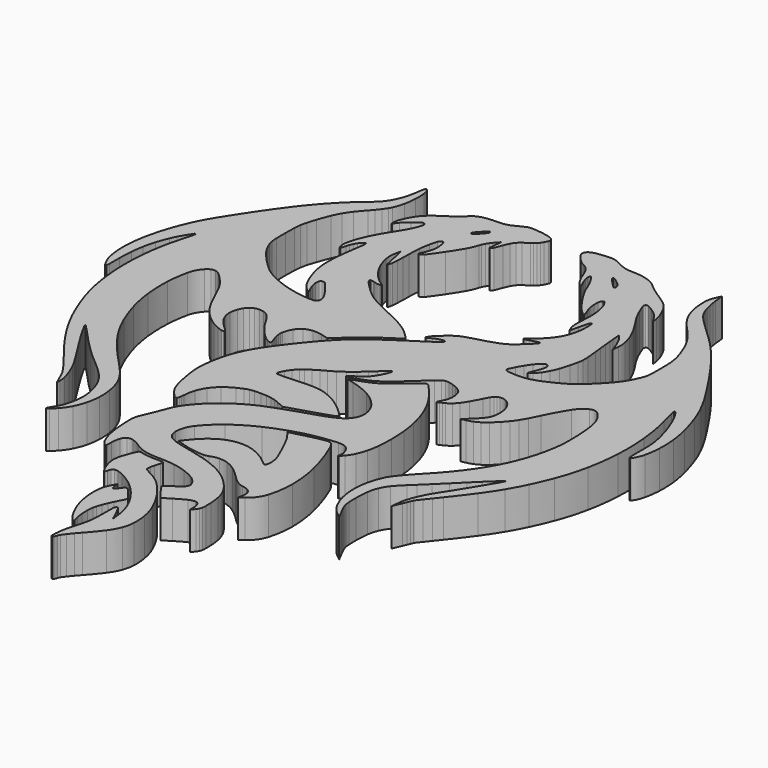
from build123d import *

# Parameters (mm, degrees)
F1_DEPTH = 25


# Not quite as in the source:
# - ends of sketch curves that miss each other by under 0.0002 mm in the source are joined


with BuildPart() as f1:
    # F0 (on Top) → F1 (new body)
    with BuildSketch(Plane.XY):
        with BuildLine():
            ThreePointArc((-98.8203232674, 222.843536045), (-99.1446126072, 220.8433618469), (-99.445342258, 218.8395100372))
            ThreePointArc((-99.445342258, 218.8395100372), (-100.0795624642, 215.3080653379), (-100.956565693, 211.8289559112))
            ThreePointArc((-100.956565693, 211.8289559112), (-102.010542388, 208.7173591719), (-103.3401926156, 205.7132068087))
            ThreePointArc((-103.3401926156, 205.7132068087), (-104.8237989366, 203.0667893306), (-106.5603216081, 200.5789986967))
            ThreePointArc((-106.5603216081, 200.5789986967), (-108.4434769256, 198.4187442732), (-110.5653861389, 196.4924851722))
            ThreePointArc((-110.5653861389, 196.4924851722), (-116.3197506967, 191.6158020551), (-121.8306110477, 186.4655430486))
            ThreePointArc((-121.8306110477, 186.4655430486), (-127.2341749271, 180.9204998118), (-132.3833899822, 175.1384939848))
            ThreePointArc((-132.3833899822, 175.1384939848), (-137.8880213543, 168.4093432424), (-143.1263111117, 161.4708450809))
            ThreePointArc((-143.1263111117, 161.4708450809), (-149.1688206673, 152.933505365), (-155.0175967206, 144.2622938161))
            ThreePointArc((-155.0175967206, 144.2622938161), (-158.9483442827, 138.2071953283), (-162.8016949017, 132.1025509388))
            ThreePointArc((-162.8016949017, 132.1025509388), (-165.3759000928, 127.7933973021), (-167.7915728682, 123.3934129307))
            ThreePointArc((-167.7915728682, 123.3934129307), (-169.719141963, 119.5124250189), (-171.4669390691, 115.5472270286))
            ThreePointArc((-171.4669390691, 115.5472270286), (-173.2388369172, 111.054752636), (-174.8608859969, 106.506026999))
            ThreePointArc((-174.8608859969, 106.506026999), (-177.1991958523, 98.7791444985), (-179.0368861575, 90.9181458314))
            ThreePointArc((-179.0368861575, 90.9181458314), (-180.1534782822, 83.7202961), (-180.6383398907, 76.4525090205))
            ThreePointArc((-180.6383398907, 76.4525090205), (-180.4661889612, 70.1986509122), (-179.6644360757, 63.9940099863))
            ThreePointArc((-179.6644360757, 63.9940099863), (-178.2981852156, 59.0735413803), (-176.0561446567, 54.4854146006))
            ThreePointArc((-176.0561446567, 54.4854146006), (-175.6038935457, 53.8635532443), (-175.0557479371, 53.3243140754))
            ThreePointArc((-175.0557479371, 53.3243140754), (-174.717000027, 53.2644494336), (-174.4938314515, 53.526231085))
            ThreePointArc((-174.4938314515, 53.526231085), (-174.3421287795, 54.5893224548), (-174.2851217529, 55.6616690066))
            ThreePointArc((-174.2851217529, 55.6616690066), (-174.2540846533, 59.9090907413), (-174.2356801238, 64.1565860004))
            ThreePointArc((-174.2356801238, 64.1565860004), (-174.1271753204, 68.7979573987), (-173.8282581789, 73.4309640152))
            ThreePointArc((-173.8282581789, 73.4309640152), (-173.3543109175, 77.6614465523), (-172.6560140174, 81.8607310034))
            ThreePointArc((-172.6560140174, 81.8607310034), (-171.7581852843, 85.8958527281), (-170.6395125581, 89.8754098625))
            ThreePointArc((-170.6395125581, 89.8754098625), (-169.2686365003, 93.9237817647), (-167.6977442352, 97.8988180998))
            ThreePointArc((-167.6977442352, 97.8988180998), (-166.8110995297, 99.8639484126), (-165.8367048947, 101.7870789436))
            ThreePointArc((-165.8367048947, 101.7870789436), (-164.6452224096, 103.9329478897), (-163.388535748, 106.0412938445))
            ThreePointArc((-163.388535748, 106.0412938445), (-162.1548359951, 108.0103144697), (-160.8941641167, 109.9621760765))
            ThreePointArc((-160.8941641167, 109.9621760765), (-160.5693387061, 110.1597590429), (-160.2110879381, 110.0324530619))
            ThreePointArc((-160.2110879381, 110.0324530619), (-160.1087364128, 109.8600200052), (-160.1014698016, 109.659629957))
            ThreePointArc((-160.1014698016, 109.659629957), (-160.3738420552, 108.4227247821), (-160.6543049868, 107.187628997))
            ThreePointArc((-160.6543049868, 107.187628997), (-161.0017472966, 105.737068599), (-161.3738833994, 104.2926461065))
            ThreePointArc((-161.3738833994, 104.2926461065), (-161.8319307867, 102.6118375397), (-162.3080132862, 100.936048083))
            ThreePointArc((-162.3080132862, 100.936048083), (-164.8204048905, 90.8275841205), (-166.5463959594, 80.5555779948))
            ThreePointArc((-166.5463959594, 80.5555779948), (-167.5403088162, 69.8640533432), (-167.7794951101, 59.1290939986))
            ThreePointArc((-167.7794951101, 59.1290939986), (-167.2646102484, 48.5218112861), (-165.9970411344, 37.977958979))
            ThreePointArc((-165.9970411344, 37.977958979), (-164.0267001203, 28.1003584503), (-161.2408187522, 18.4210970826))
            ThreePointArc((-161.2408187522, 18.4210970826), (-158.4021079817, 10.5040916002), (-155.2123317189, 2.7218951226))
            ThreePointArc((-155.2123317189, 2.7218951226), (-151.8521030275, -4.4508084625), (-148.1130054689, -11.4334986971))
            ThreePointArc((-148.1130054689, -11.4334986971), (-143.7570895136, -18.6502392725), (-139.050614265, -25.643410188))
            ThreePointArc((-139.050614265, -25.643410188), (-133.1545970578, -33.6964505863), (-127.0207666726, -41.569861737))
            ThreePointArc((-127.0207666726, -41.569861737), (-125.192604593, -43.8790619962), (-123.3974992617, -46.2140521982))
            ThreePointArc((-123.3974992617, -46.2140521982), (-121.699811115, -48.492461708), (-120.0384609136, -50.7975019388))
            ThreePointArc((-120.0384609136, -50.7975019388), (-118.653662202, -52.782297779), (-117.2984087362, -54.7873838246))
            ThreePointArc((-117.2984087362, -54.7873838246), (-116.6201672032, -55.9029054869), (-116.0348359708, -57.0698619868))
            ThreePointArc((-116.0348359708, -57.0698619868), (-115.6332728977, -57.9592624214), (-115.2319456951, -58.8487693135))
            ThreePointArc((-115.2319456951, -58.8487693135), (-114.8038455779, -59.7982263817), (-114.3759530739, -60.7477770333))
            ThreePointArc((-114.3759530739, -60.7477770333), (-113.9831651289, -61.6199353858), (-113.590570071, -62.492180582))
            ThreePointArc((-113.590570071, -62.492180582), (-113.3106065578, -63.1148613116), (-113.0310075273, -63.737705788))
            Line((-113.0310075273, -63.737705788), (-111.909623, -66.237706))
            Line((-111.909623, -66.237706), (-111.841942, -63.593041))
            ThreePointArc((-111.841942, -63.593041), (-111.939235828, -61.4554765144), (-112.3383601064, -59.3532520281))
            ThreePointArc((-112.3383601064, -59.3532520281), (-113.2133716441, -56.3358124462), (-114.2294673716, -53.3629121369))
            ThreePointArc((-114.2294673716, -53.3629121369), (-115.5049041187, -50.1342544253), (-116.9295650629, -46.9686090301))
            ThreePointArc((-116.9295650629, -46.9686090301), (-118.4225440186, -44.0592513244), (-120.0754898718, -41.23770592))
            ThreePointArc((-120.0754898718, -41.23770592), (-121.1304904051, -39.5480863319), (-122.1866021758, -37.85916111))
            ThreePointArc((-122.1866021758, -37.85916111), (-123.587041062, -35.6219410978), (-124.9881246925, -33.3851248073))
            ThreePointArc((-124.9881246925, -33.3851248073), (-126.4757633264, -31.0116368476), (-127.9640802048, -28.6385741285))
            ThreePointArc((-127.9640802048, -28.6385741285), (-129.3146835511, -26.4866809646), (-130.6661090135, -24.3353040085))
            ThreePointArc((-130.6661090135, -24.3353040085), (-132.6969217836, -21.0703464833), (-134.6974540214, -17.7867480129))
            ThreePointArc((-134.6974540214, -17.7867480129), (-136.3342092237, -15.0230038756), (-137.9271628321, -12.2337839059))
            ThreePointArc((-137.9271628321, -12.2337839059), (-139.1916656607, -9.9532345871), (-140.4344510589, -7.6607780316))
            ThreePointArc((-140.4344510589, -7.6607780316), (-140.6880105391, -7.0051349094), (-140.774262, -6.307481))
            ThreePointArc((-140.774262, -6.307481), (-140.7237875565, -6.2324968102), (-140.6353201647, -6.2510391602))
            ThreePointArc((-140.6353201647, -6.2510391602), (-139.254639861, -7.672491093), (-137.8764750026, -9.0963820026))
            ThreePointArc((-137.8764750026, -9.0963820026), (-136.2783350371, -10.7632913491), (-134.6931009877, -12.4424789884))
            ThreePointArc((-134.6931009877, -12.4424789884), (-132.7967478611, -14.475855389), (-130.9094539043, -16.5176429119))
            ThreePointArc((-130.9094539043, -16.5176429119), (-128.7516998845, -18.8251103941), (-126.5572687318, -21.0977257368))
            ThreePointArc((-126.5572687318, -21.0977257368), (-124.1092876703, -23.56273749), (-121.631772005, -25.9980630052))
            ThreePointArc((-121.631772005, -25.9980630052), (-119.2733065512, -28.260809788), (-116.8874295002, -30.4946345409))
            ThreePointArc((-116.8874295002, -30.4946345409), (-115.0556228293, -32.1420455045), (-113.1785655234, -33.7377066334))
            ThreePointArc((-113.1785655234, -33.7377066334), (-108.1269376279, -38.0604455111), (-103.2270552204, -42.5544602322))
            ThreePointArc((-103.2270552204, -42.5544602322), (-100.1049452848, -45.8422541348), (-97.3396797067, -49.4353677975))
            ThreePointArc((-97.3396797067, -49.4353677975), (-95.3307810205, -52.7995537807), (-93.7807023803, -56.3982587802))
            ThreePointArc((-93.7807023803, -56.3982587802), (-92.4508001025, -60.7265979852), (-91.4959783635, -65.152823891))
            ThreePointArc((-91.4959783635, -65.152823891), (-91.1473268936, -68.1147781546), (-91.1108842268, -71.0969589909))
            ThreePointArc((-91.1108842268, -71.0969589909), (-91.3724825494, -74.3596281344), (-91.892383303, -77.5912139388))
            ThreePointArc((-91.892383303, -77.5912139388), (-92.6608735665, -80.7411014363), (-93.6788362236, -83.8194322917))
            ThreePointArc((-93.6788362236, -83.8194322917), (-94.8466039887, -86.4648800928), (-96.3042316862, -88.9623582077))
            ThreePointArc((-96.3042316862, -88.9623582077), (-97.2655022272, -90.4794950758), (-98.1658367809, -92.0335681212))
            ThreePointArc((-98.1658367809, -92.0335681212), (-98.1434567179, -92.4336210577), (-97.7732690816, -92.5869325203))
            ThreePointArc((-97.7732690816, -92.5869325203), (-96.9964744052, -92.3270823597), (-96.3353206325, -91.8435453672))
            ThreePointArc((-96.3353206325, -91.8435453672), (-94.6686599424, -90.1416500982), (-93.0366306778, -88.406517297))
            ThreePointArc((-93.0366306778, -88.406517297), (-90.5707409165, -85.3312318156), (-88.5503146074, -81.946579692))
            ThreePointArc((-88.5503146074, -81.946579692), (-86.8363121326, -78.0513485831), (-85.5585530156, -73.992042996))
            ThreePointArc((-85.5585530156, -73.992042996), (-84.6800586672, -69.6135822051), (-84.2622427468, -65.167448969))
            ThreePointArc((-84.2622427468, -65.167448969), (-84.3005019897, -60.6380683498), (-84.7906495928, -56.135123935))
            ThreePointArc((-84.7906495928, -56.135123935), (-85.5630774303, -52.296694583), (-86.6410640206, -48.5326370068))
            ThreePointArc((-86.6410640206, -48.5326370068), (-87.9268442538, -45.2615106235), (-89.5665778482, -42.1526889089))
            ThreePointArc((-89.5665778482, -42.1526889089), (-91.8631743382, -38.669024401), (-94.4443773043, -35.390661261))
            ThreePointArc((-94.4443773043, -35.390661261), (-98.5395630445, -30.7455515771), (-102.7588696488, -26.2128876641))
            ThreePointArc((-102.7588696488, -26.2128876641), (-108.6377698425, -19.8010841412), (-114.2414051391, -13.1473661122))
            ThreePointArc((-114.2414051391, -13.1473661122), (-118.7174977583, -7.2022861768), (-122.785357815, -0.9707618879))
            ThreePointArc((-122.785357815, -0.9707618879), (-126.2214440317, 5.1884428501), (-129.2062188958, 11.5785610442))
            ThreePointArc((-129.2062188958, 11.5785610442), (-131.9323675691, 18.580455177), (-134.2374512463, 25.7320282184))
            ThreePointArc((-134.2374512463, 25.7320282184), (-136.2041868479, 33.7774706829), (-137.4838796257, 41.9603540424))
            ThreePointArc((-137.4838796257, 41.9603540424), (-138.0969447424, 50.3724153506), (-138.0346620567, 58.8065570027))
            ThreePointArc((-138.0346620567, 58.8065570027), (-137.3753464853, 66.1376764758), (-136.0998020812, 73.3870210178))
            ThreePointArc((-136.0998020812, 73.3870210178), (-134.4143809266, 77.992035102), (-131.5661473718, 81.9838223493))
            ThreePointArc((-131.5661473718, 81.9838223493), (-130.3000205965, 83.0868574718), (-128.8400928888, 83.9165407488))
            ThreePointArc((-128.8400928888, 83.9165407488), (-127.4707488648, 84.2691021796), (-126.0610140725, 84.1593277071))
            ThreePointArc((-126.0610140725, 84.1593277071), (-124.4164851324, 83.5479804552), (-122.9514408764, 82.5826481479))
            ThreePointArc((-122.9514408764, 82.5826481479), (-120.9740909201, 80.8105163837), (-119.1246050846, 78.9053219234))
            ThreePointArc((-119.1246050846, 78.9053219234), (-117.4547800909, 76.9992962406), (-115.8482208797, 75.0396490954))
            ThreePointArc((-115.8482208797, 75.0396490954), (-114.6698583722, 73.4457766834), (-113.6015905792, 71.7761146564))
            ThreePointArc((-113.6015905792, 71.7761146564), (-112.4130189266, 69.6653889442), (-111.3210566937, 67.5031021461))
            ThreePointArc((-111.3210566937, 67.5031021461), (-109.3795797156, 63.3903730479), (-107.4709582702, 59.2622938764))
            ThreePointArc((-107.4709582702, 59.2622938764), (-105.8977018573, 55.9935562367), (-104.1982675448, 52.7886062529))
            ThreePointArc((-104.1982675448, 52.7886062529), (-102.6267256736, 50.1630204129), (-100.8889277339, 47.6443891966))
            ThreePointArc((-100.8889277339, 47.6443891966), (-99.116356377, 45.4150158059), (-97.1902278217, 43.3168871757))
            ThreePointArc((-97.1902278217, 43.3168871757), (-95.0328531717, 41.2593910555), (-92.7523819261, 39.3392330934))
            ThreePointArc((-92.7523819261, 39.3392330934), (-90.9357531207, 38.000005137), (-89.0332178483, 36.7859082564))
            ThreePointArc((-89.0332178483, 36.7859082564), (-87.0413341844, 35.6941800348), (-84.9818027965, 34.7361604781))
            ThreePointArc((-84.9818027965, 34.7361604781), (-83.206138052, 34.0420505443), (-81.3923248496, 33.4548065164))
            ThreePointArc((-81.3923248496, 33.4548065164), (-80.5691273826, 33.4415001977), (-79.8539170773, 33.8493060773))
            ThreePointArc((-79.8539170773, 33.8493060773), (-79.7718184632, 34.0257296141), (-79.8226271048, 34.2135699261))
            ThreePointArc((-79.8226271048, 34.2135699261), (-80.1783332955, 34.6959473687), (-80.5543244981, 35.1626865809))
            ThreePointArc((-80.5543244981, 35.1626865809), (-81.0730020421, 35.7496324041), (-81.6195080954, 36.3107589025))
            ThreePointArc((-81.6195080954, 36.3107589025), (-82.2938154198, 36.9514220509), (-82.986471896, 37.5722011195))
            ThreePointArc((-82.986471896, 37.5722011195), (-85.2798438969, 39.7821885927), (-87.3377148259, 42.2129841328))
            ThreePointArc((-87.3377148259, 42.2129841328), (-88.8200239087, 44.5137654092), (-89.9194801991, 47.0201632778))
            ThreePointArc((-89.9194801991, 47.0201632778), (-90.5249213408, 49.4496882645), (-90.6872031185, 51.9482510029))
            ThreePointArc((-90.6872031185, 51.9482510029), (-90.408730088, 54.4891278609), (-89.7076506726, 56.9471942548))
            ThreePointArc((-89.7076506726, 56.9471942548), (-88.9973959277, 58.5623625708), (-88.1229624952, 60.094875676))
            ThreePointArc((-88.1229624952, 60.094875676), (-87.1920267741, 61.3233544423), (-86.0818556516, 62.3926165769))
            ThreePointArc((-86.0818556516, 62.3926165769), (-84.9146190025, 63.193968172), (-83.6261000142, 63.7807600402))
            ThreePointArc((-83.6261000142, 63.7807600402), (-82.2448028738, 64.1410352346), (-80.822454, 64.262294))
            ThreePointArc((-80.822454, 64.262294), (-79.1611459359, 64.1460661058), (-77.5322049722, 63.7996490969))
            ThreePointArc((-77.5322049722, 63.7996490969), (-76.1410958268, 63.2512099916), (-74.8804377595, 62.4470263073))
            ThreePointArc((-74.8804377595, 62.4470263073), (-73.5570883187, 61.2479308782), (-72.4200717174, 59.8708772009))
            ThreePointArc((-72.4200717174, 59.8708772009), (-70.9706107086, 57.7215999972), (-69.6289158046, 55.5034511117))
            ThreePointArc((-69.6289158046, 55.5034511117), (-68.0955582073, 52.9809617849), (-66.4289372996, 50.544465783))
            ThreePointArc((-66.4289372996, 50.544465783), (-64.5878976774, 48.1301436754), (-62.6299088027, 45.809657175))
            ThreePointArc((-62.6299088027, 45.809657175), (-60.7640756053, 43.8116212623), (-58.7983248161, 41.9118042003))
            ThreePointArc((-58.7983248161, 41.9118042003), (-57.2620655648, 40.6787402695), (-55.5761311444, 39.6598367208))
            ThreePointArc((-55.5761311444, 39.6598367208), (-54.5843229691, 39.1818077356), (-53.5672099095, 38.760291237))
            ThreePointArc((-53.5672099095, 38.760291237), (-53.2015160144, 38.7792884643), (-52.9696765803, 39.0627378843))
            ThreePointArc((-52.9696765803, 39.0627378843), (-52.9007814903, 39.6182950807), (-52.9942134887, 40.1702558417))
            ThreePointArc((-52.9942134887, 40.1702558417), (-53.6538995331, 42.1697238529), (-54.3354205576, 44.1618551541))
            ThreePointArc((-54.3354205576, 44.1618551541), (-54.6515563694, 45.1554487853), (-54.9135005866, 46.1646838646))
            ThreePointArc((-54.9135005866, 46.1646838646), (-55.1185337851, 47.1798530959), (-55.2672401399, 48.2047889836))
            ThreePointArc((-55.2672401399, 48.2047889836), (-55.3498978352, 49.1516458399), (-55.3767615558, 50.1017239995))
            ThreePointArc((-55.3767615558, 50.1017239995), (-55.3352636914, 50.8860288153), (-55.2129941762, 51.6618550372))
            ThreePointArc((-55.2129941762, 51.6618550372), (-54.3225687778, 54.6559929347), (-52.9607453022, 57.4672481779))
            ThreePointArc((-52.9607453022, 57.4672481779), (-51.3080221726, 59.6200039237), (-49.1820783394, 61.3070765559))
            ThreePointArc((-49.1820783394, 61.3070765559), (-46.6949198577, 62.4381480307), (-44.0088060151, 62.9382202407))
            ThreePointArc((-44.0088060151, 62.9382202407), (-40.8400277143, 62.8884467812), (-37.717890937, 62.3444842458))
            Line((-37.717890937, 62.3444842458), (-32.772195, 61.07694))
            Line((-32.772195, 61.07694), (-25.695259, 67.629098))
            ThreePointArc((-25.695259, 67.629098), (-24.0476694838, 69.1143352019), (-22.3611827957, 70.5552527543))
            ThreePointArc((-22.3611827957, 70.5552527543), (-20.2680089465, 72.2700869555), (-18.149763709, 73.9538536283))
            ThreePointArc((-18.149763709, 73.9538536283), (-15.9776155749, 75.6288581524), (-13.7810745195, 77.2717443477))
            ThreePointArc((-13.7810745195, 77.2717443477), (-11.8795048237, 78.6380875895), (-9.9462918103, 79.9592797152))
            ThreePointArc((-9.9462918103, 79.9592797152), (-8.2661949875, 81.0791655638), (-6.5865280675, 82.1996961012))
            ThreePointArc((-6.5865280675, 82.1996961012), (-5.1303764038, 83.1721391155), (-3.6747964281, 84.1454376398))
            ThreePointArc((-3.6747964281, 84.1454376398), (-2.4159482812, 84.9878999239), (-1.1572658546, 85.8306097829))
            ThreePointArc((-1.1572658546, 85.8306097829), (-0.9646845929, 85.9618524476), (-0.7742618447, 86.0962077837))
            ThreePointArc((-0.7742618447, 86.0962077837), (-0.691585246, 86.236463494), (-0.7394655437, 86.3920735288))
            ThreePointArc((-0.7394655437, 86.3920735288), (-1.3622607438, 87.1006094038), (-1.9949340277, 87.8003389746))
            ThreePointArc((-1.9949340277, 87.8003389746), (-2.7929750971, 88.6478357024), (-3.6131547066, 89.4739262992))
            ThreePointArc((-3.6131547066, 89.4739262992), (-4.6150599091, 90.4415548935), (-5.6318682342, 91.3935107459))
            ThreePointArc((-5.6318682342, 91.3935107459), (-7.093046229, 92.6655459779), (-8.6240742385, 93.8525876737))
            ThreePointArc((-8.6240742385, 93.8525876737), (-10.4522983097, 95.1373203172), (-12.326948765, 96.3533083775))
            ThreePointArc((-12.326948765, 96.3533083775), (-14.4805387571, 97.6449326992), (-16.6758653458, 98.8642703523))
            ThreePointArc((-16.6758653458, 98.8642703523), (-19.1384869935, 100.1401690562), (-21.6318678872, 101.3548602389))
            ThreePointArc((-21.6318678872, 101.3548602389), (-28.1264670157, 104.4443544516), (-34.6021431345, 107.5733177237))
            ThreePointArc((-34.6021431345, 107.5733177237), (-37.7249125081, 109.1770289585), (-40.7766148355, 110.9121632756))
            ThreePointArc((-40.7766148355, 110.9121632756), (-43.0269217614, 112.3703936748), (-45.1642298616, 113.9897241694))
            ThreePointArc((-45.1642298616, 113.9897241694), (-47.6331174182, 116.094463347), (-50.012041764, 118.3003762441))
            ThreePointArc((-50.012041764, 118.3003762441), (-52.3320573716, 120.5889364484), (-54.6057252167, 122.9235487932))
            ThreePointArc((-54.6057252167, 122.9235487932), (-55.6287212533, 124.1549515548), (-56.4727779779, 125.5152610117))
            ThreePointArc((-56.4727779779, 125.5152610117), (-56.4830615536, 126.065674741), (-56.0461480406, 126.4005892154))
            ThreePointArc((-56.0461480406, 126.4005892154), (-55.1163828612, 126.4460653072), (-54.2091618886, 126.2375432929))
            ThreePointArc((-54.2091618886, 126.2375432929), (-53.6429278083, 126.0383570877), (-53.0674230041, 125.8677979849))
            ThreePointArc((-53.0674230041, 125.8677979849), (-52.4142859025, 125.7043189837), (-51.7557461002, 125.564180484))
            ThreePointArc((-51.7557461002, 125.564180484), (-51.1194357387, 125.452421792), (-50.4795119628, 125.3636613087))
            ThreePointArc((-50.4795119628, 125.3636613087), (-49.9702166966, 125.320853324), (-49.4591619949, 125.3147457884))
            ThreePointArc((-49.4591619949, 125.3147457884), (-48.7630826694, 125.338730542), (-48.0676559738, 125.3772456018))
            ThreePointArc((-48.0676559738, 125.3772456018), (-47.9400301643, 125.4448722929), (-47.9056223658, 125.5851499331))
            ThreePointArc((-47.9056223658, 125.5851499331), (-47.9782147176, 125.7683611516), (-48.1153748372, 125.9098642356))
            ThreePointArc((-48.1153748372, 125.9098642356), (-48.9425863321, 126.4766814517), (-49.7742619832, 127.0369280252))
            ThreePointArc((-49.7742619832, 127.0369280252), (-53.4600020251, 129.8989589134), (-56.7008866701, 133.2564232758))
            ThreePointArc((-56.7008866701, 133.2564232758), (-59.6076884755, 137.2041155058), (-62.0070590794, 141.4792519617))
            ThreePointArc((-62.0070590794, 141.4792519617), (-63.7594113069, 145.800348757), (-64.9410622105, 150.3110379591))
            ThreePointArc((-64.9410622105, 150.3110379591), (-65.3089104498, 154.3144809668), (-64.8736434599, 158.3111558857))
            Line((-64.8736434599, 158.3111558857), (-64.143351, 161.762294))
            Line((-64.143351, 161.762294), (-63.00649, 156.762294))
            ThreePointArc((-63.00649, 156.762294), (-62.761252797, 155.6774169652), (-62.5187433721, 154.5919269174))
            ThreePointArc((-62.5187433721, 154.5919269174), (-62.2546937377, 153.3976717789), (-61.992904739, 152.2029190569))
            ThreePointArc((-61.992904739, 152.2029190569), (-61.748872249, 151.0789796696), (-61.5069884565, 149.9545759022))
            ThreePointArc((-61.5069884565, 149.9545759022), (-61.3278450012, 149.1088257425), (-61.1524327411, 148.2622938481))
            ThreePointArc((-61.1524327411, 148.2622938481), (-60.911623616, 147.1053613181), (-60.6636512824, 145.9499429385))
            ThreePointArc((-60.6636512824, 145.9499429385), (-60.5811710499, 145.756202216), (-60.4333189977, 145.6062750033))
            ThreePointArc((-60.4333189977, 145.6062750033), (-60.2928081856, 145.5864969562), (-60.1928601586, 145.687218052))
            ThreePointArc((-60.1928601586, 145.687218052), (-59.9422261994, 146.4727658363), (-59.704428632, 147.2622941848))
            ThreePointArc((-59.704428632, 147.2622941848), (-59.5174526505, 148.0471695374), (-59.410623345, 148.8469050284))
            ThreePointArc((-59.410623345, 148.8469050284), (-59.2681802252, 150.6991833842), (-59.1461577949, 152.5529189876))
            ThreePointArc((-59.1461577949, 152.5529189876), (-59.0275064981, 154.7678947353), (-58.9385581489, 156.984262005))
            ThreePointArc((-58.9385581489, 156.984262005), (-58.8715532053, 159.3729873742), (-58.8301724978, 161.762294006))
            ThreePointArc((-58.8301724978, 161.762294006), (-58.7035487419, 165.9539216912), (-58.4240825415, 170.1381390461))
            ThreePointArc((-58.4240825415, 170.1381390461), (-58.0180254705, 173.6334867564), (-57.3981491661, 177.0973128242))
            ThreePointArc((-57.3981491661, 177.0973128242), (-56.7605971955, 179.6919954805), (-55.9525643682, 182.2387451304))
            ThreePointArc((-55.9525643682, 182.2387451304), (-55.2537175569, 183.3266305065), (-54.1437159168, 183.9897877382))
            ThreePointArc((-54.1437159168, 183.9897877382), (-53.5288850678, 183.9435110015), (-53.1178924268, 183.4838988458))
            ThreePointArc((-53.1178924268, 183.4838988458), (-52.6760657969, 182.077708054), (-52.3541959277, 180.639312013))
            ThreePointArc((-52.3541959277, 180.639312013), (-52.1122364195, 178.8807087919), (-52.0160924764, 177.1081439938))
            ThreePointArc((-52.0160924764, 177.1081439938), (-52.0853830356, 175.5093620623), (-52.3336588559, 173.928455969))
            ThreePointArc((-52.3336588559, 173.928455969), (-52.5010507253, 173.2188819133), (-52.6962123063, 172.5164380916))
            ThreePointArc((-52.6962123063, 172.5164380916), (-52.9520977976, 171.6972715469), (-53.2277428083, 170.8845409324))
            ThreePointArc((-53.2277428083, 170.8845409324), (-53.5205164098, 170.0855340057), (-53.8325936073, 169.293867248))
            ThreePointArc((-53.8325936073, 169.293867248), (-54.1129044642, 168.6468511672), (-54.4203800548, 168.012294028))
            ThreePointArc((-54.4203800548, 168.012294028), (-54.6724514401, 167.4901071768), (-54.9005892463, 166.9570290989))
            ThreePointArc((-54.9005892463, 166.9570290989), (-55.0543263571, 166.5194578737), (-55.1691636538, 166.0701071369))
            ThreePointArc((-55.1691636538, 166.0701071369), (-55.2110248352, 165.7680710883), (-55.2111541789, 165.4631480561))
            ThreePointArc((-55.2111541789, 165.4631480561), (-55.1432370239, 165.3203174285), (-54.996109, 165.262294))
            ThreePointArc((-54.996109, 165.262294), (-53.4048326662, 165.6405965789), (-52.1540549066, 166.6945549308))
            ThreePointArc((-52.1540549066, 166.6945549308), (-48.8178993391, 171.3022914388), (-45.5793528001, 175.9791478647))
            ThreePointArc((-45.5793528001, 175.9791478647), (-42.4868955516, 180.7256415091), (-39.5642807353, 185.5785598469))
            ThreePointArc((-39.5642807353, 185.5785598469), (-37.8864249646, 188.9141834661), (-36.608146826, 192.4224009479))
            ThreePointArc((-36.608146826, 192.4224009479), (-36.3183572485, 193.2746659888), (-35.9669116817, 194.103411851))
            ThreePointArc((-35.9669116817, 194.103411851), (-35.4819157204, 195.0867967391), (-34.9571304526, 196.0495362589))
            ThreePointArc((-34.9571304526, 196.0495362589), (-34.382141594, 197.0091693302), (-33.768676612, 197.9446737342))
            ThreePointArc((-33.768676612, 197.9446737342), (-33.1947352094, 198.7292803015), (-32.5735113289, 199.4770082909))
            Line((-32.5735113289, 199.4770082909), (-29.668192, 202.762294))
            Line((-29.668192, 202.762294), (-30.298513, 197.905512))
            ThreePointArc((-30.298513, 197.905512), (-30.4965619638, 196.0463573022), (-30.6091564475, 194.1800770167))
            ThreePointArc((-30.6091564475, 194.1800770167), (-30.385533678, 193.7826264518), (-29.929881755, 193.801474635))
            ThreePointArc((-29.929881755, 193.801474635), (-29.2457725018, 194.422773426), (-28.7697206373, 195.2148542657))
            ThreePointArc((-28.7697206373, 195.2148542657), (-27.7462993407, 197.7351905327), (-26.7698488339, 200.2740939379))
            ThreePointArc((-26.7698488339, 200.2740939379), (-25.96834694, 202.247686504), (-25.058046996, 204.173517998))
            ThreePointArc((-25.058046996, 204.173517998), (-24.236365103, 205.5711329138), (-23.2480252955, 206.8563072579))
            ThreePointArc((-23.2480252955, 206.8563072579), (-22.100003841, 208.0195131105), (-20.8185196101, 209.0338104402))
            ThreePointArc((-20.8185196101, 209.0338104402), (-19.0010602753, 210.2291957301), (-17.1227465967, 211.3264842655))
            ThreePointArc((-17.1227465967, 211.3264842655), (-16.4827778097, 211.7242004816), (-15.8892913838, 212.1884332941))
            ThreePointArc((-15.8892913838, 212.1884332941), (-15.1922869386, 212.8313341855), (-14.5314911974, 213.5113971816))
            ThreePointArc((-14.5314911974, 213.5113971816), (-13.877850811, 214.2614130926), (-13.2653648828, 215.0453969134))
            ThreePointArc((-13.2653648828, 215.0453969134), (-12.7559955899, 215.7893238615), (-12.3014503141, 216.5679591685))
            ThreePointArc((-12.3014503141, 216.5679591685), (-11.7314922432, 217.6636354616), (-11.1896397131, 218.7734798644))
            ThreePointArc((-11.1896397131, 218.7734798644), (-10.9865294815, 219.331153383), (-10.8890685873, 219.9166060428))
            ThreePointArc((-10.8890685873, 219.9166060428), (-10.9277699817, 220.3795682849), (-11.1068889644, 220.8082270219))
            ThreePointArc((-11.1068889644, 220.8082270219), (-11.4821910013, 221.3447933975), (-11.9174126349, 221.8340143651))
            ThreePointArc((-11.9174126349, 221.8340143651), (-12.4249734926, 222.2441234591), (-13.0073477805, 222.5384835792))
            ThreePointArc((-13.0073477805, 222.5384835792), (-14.0715615385, 222.9140109061), (-15.151896826, 223.240273628))
            ThreePointArc((-15.151896826, 223.240273628), (-16.5091830682, 223.5848208109), (-17.8801539016, 223.8700885304))
            ThreePointArc((-17.8801539016, 223.8700885304), (-19.4439334002, 224.1360253529), (-21.0149759784, 224.3550091743))
            ThreePointArc((-21.0149759784, 224.3550091743), (-23.3781134496, 224.6231475821), (-25.746375953, 224.8414355768))
            ThreePointArc((-25.746375953, 224.8414355768), (-27.0158526274, 224.8694432165), (-28.2797210148, 224.7470010945))
            ThreePointArc((-28.2797210148, 224.7470010945), (-29.4570860105, 224.480478655), (-30.5885210028, 224.0596730063))
            ThreePointArc((-30.5885210028, 224.0596730063), (-32.4332537819, 223.1953525572), (-34.2505597994, 222.2747616187))
            ThreePointArc((-34.2505597994, 222.2747616187), (-35.8844411343, 221.4563402119), (-37.549564959, 220.7035159044))
            ThreePointArc((-37.549564959, 220.7035159044), (-38.8630844916, 220.2066050991), (-40.2144807751, 219.8245290501))
            ThreePointArc((-40.2144807751, 219.8245290501), (-41.6291043538, 219.5506800437), (-43.0614840343, 219.3943425072))
            ThreePointArc((-43.0614840343, 219.3943425072), (-45.0169678728, 219.2953160629), (-46.974679, 219.262294))
            ThreePointArc((-46.974679, 219.262294), (-49.6014150187, 219.1770442219), (-52.2170960056, 218.9216570427))
            ThreePointArc((-52.2170960056, 218.9216570427), (-54.444582281, 218.5156137855), (-56.6197298883, 217.886885676))
            ThreePointArc((-56.6197298883, 217.886885676), (-58.3545006397, 217.1665076892), (-59.9874611469, 216.2381682249))
            ThreePointArc((-59.9874611469, 216.2381682249), (-61.1729259617, 215.2600528465), (-62.1133459793, 214.0444679874))
            ThreePointArc((-62.1133459793, 214.0444679874), (-62.4797197332, 213.5365370688), (-62.9202686711, 213.0914076196))
            ThreePointArc((-62.9202686711, 213.0914076196), (-63.7974129004, 212.355219078), (-64.6957431264, 211.6450371648))
            ThreePointArc((-64.6957431264, 211.6450371648), (-65.7817931681, 210.838168167), (-66.8920859291, 210.0649978948))
            ThreePointArc((-66.8920859291, 210.0649978948), (-68.0729426088, 209.2923199627), (-69.2742617164, 208.5518565256))
            ThreePointArc((-69.2742617164, 208.5518565256), (-70.5751160432, 207.7506693791), (-71.854414131, 206.9154931949))
            ThreePointArc((-71.854414131, 206.9154931949), (-73.260700677, 205.9512736162), (-74.6484369125, 204.9605418799))
            ThreePointArc((-74.6484369125, 204.9605418799), (-75.9519132696, 203.9918936795), (-77.2365649403, 202.9984149243))
            ThreePointArc((-77.2365649403, 202.9984149243), (-78.2068629733, 202.2004034174), (-79.1437936501, 201.363467624))
            ThreePointArc((-79.1437936501, 201.363467624), (-80.8234403154, 199.6337801111), (-82.3198121031, 197.7433030735))
            ThreePointArc((-82.3198121031, 197.7433030735), (-83.8083913657, 195.4861939984), (-85.1310138398, 193.1279999176))
            ThreePointArc((-85.1310138398, 193.1279999176), (-86.2088760817, 190.8301789392), (-87.1158268614, 188.4596919527))
            ThreePointArc((-87.1158268614, 188.4596919527), (-87.563736221, 186.6361167525), (-87.6855460477, 184.7622939989))
            ThreePointArc((-87.6855460477, 184.7622939989), (-87.6642558651, 184.2269225358), (-87.6251083179, 183.6925599714))
            ThreePointArc((-87.6251083179, 183.6925599714), (-87.5737391565, 183.3828325934), (-87.4769407744, 183.0841690922))
            ThreePointArc((-87.4769407744, 183.0841690922), (-87.3945005813, 183.0059630491), (-87.2813121176, 183.0160112091))
            ThreePointArc((-87.2813121176, 183.0160112091), (-87.1548187659, 183.1204100343), (-87.0725472561, 183.2622940929))
            ThreePointArc((-87.0725472561, 183.2622940929), (-86.2317544726, 184.9887148683), (-85.0483399793, 186.50099498))
            ThreePointArc((-85.0483399793, 186.50099498), (-82.8854739377, 188.6074711484), (-80.6033162198, 190.5840812693))
            ThreePointArc((-80.6033162198, 190.5840812693), (-78.2999258683, 192.3772823315), (-75.9162750814, 194.062330121))
            ThreePointArc((-75.9162750814, 194.062330121), (-74.9565584597, 194.3052024229), (-74.0612930862, 193.8826589138))
            ThreePointArc((-74.0612930862, 193.8826589138), (-73.5960862173, 193.0894210146), (-73.5772999704, 192.1700239929))
            ThreePointArc((-73.5772999704, 192.1700239929), (-74.1023904285, 190.2572517682), (-74.7538334833, 188.3837418008))
            ThreePointArc((-74.7538334833, 188.3837418008), (-75.7573229692, 186.0098551662), (-76.910319667, 183.7048763607))
            ThreePointArc((-76.910319667, 183.7048763607), (-78.3797161268, 181.1181773345), (-79.9555940928, 178.5949360607))
            ThreePointArc((-79.9555940928, 178.5949360607), (-83.1920714706, 173.4268967259), (-86.2234166864, 168.1359268284))
            ThreePointArc((-86.2234166864, 168.1359268284), (-88.4801300635, 163.6472857424), (-90.4191112435, 159.012525092))
            ThreePointArc((-90.4191112435, 159.012525092), (-91.6448414519, 155.2941566209), (-92.5466976438, 151.4842571234))
            ThreePointArc((-92.5466976438, 151.4842571234), (-92.7231101594, 148.7843849742), (-92.2303703368, 146.1240018931))
            ThreePointArc((-92.2303703368, 146.1240018931), (-92.0300409588, 145.5823809703), (-91.7798265094, 145.061921725))
            ThreePointArc((-91.7798265094, 145.061921725), (-91.601071369, 144.9445680092), (-91.4048436242, 145.0295377038))
            ThreePointArc((-91.4048436242, 145.0295377038), (-91.1640268196, 145.4070472998), (-91.0026218338, 145.8247249541))
            ThreePointArc((-91.0026218338, 145.8247249541), (-90.6248614274, 147.221786893), (-90.2614884157, 148.6226598516))
            ThreePointArc((-90.2614884157, 148.6226598516), (-89.9633514944, 149.6552464257), (-89.5989170501, 150.6663390199))
            ThreePointArc((-89.5989170501, 150.6663390199), (-89.1368954588, 151.7499756787), (-88.6220322698, 152.8095266227))
            ThreePointArc((-88.6220322698, 152.8095266227), (-88.0855422003, 153.7865648067), (-87.5005589161, 154.7353639453))
            ThreePointArc((-87.5005589161, 154.7353639453), (-86.9874642402, 155.4396709107), (-86.4041149222, 156.0869869222))
            ThreePointArc((-86.4041149222, 156.0869869222), (-85.5616457231, 156.8386361379), (-84.6392589793, 157.4897379669))
            ThreePointArc((-84.6392589793, 157.4897379669), (-84.1933859588, 157.5134634148), (-83.9358567158, 157.1487110314))
            ThreePointArc((-83.9358567158, 157.1487110314), (-83.8824767622, 156.0483994991), (-83.9649294991, 154.9498839311))
            ThreePointArc((-83.9649294991, 154.9498839311), (-84.6051142456, 150.3549105003), (-85.2619931707, 145.7622938798))
            ThreePointArc((-85.2619931707, 145.7622938798), (-85.9035980723, 140.8415404492), (-86.4049459165, 135.9045249927))
            ThreePointArc((-86.4049459165, 135.9045249927), (-86.6475347985, 131.8938446034), (-86.6768125509, 127.8759410087))
            ThreePointArc((-86.6768125509, 127.8759410087), (-86.4998114083, 124.417926253), (-86.1029313286, 120.9782050992))
            ThreePointArc((-86.1029313286, 120.9782050992), (-85.5033365675, 117.770481791), (-84.6615996964, 114.6176287854))
            ThreePointArc((-84.6615996964, 114.6176287854), (-83.6883053655, 111.6150023138), (-82.6282570169, 108.6418953667))
            ThreePointArc((-82.6282570169, 108.6418953667), (-81.7116407309, 106.4039512661), (-80.6549598999, 104.2286340526))
            ThreePointArc((-80.6549598999, 104.2286340526), (-79.6299864051, 102.4527701889), (-78.467902103, 100.763443923))
            ThreePointArc((-78.467902103, 100.763443923), (-77.1996218079, 99.2088365945), (-75.8047805865, 97.7667004352))
            Line((-75.8047805865, 97.7667004352), (-72.652135, 94.771106))
            Line((-72.652135, 94.771106), (-74.691236, 99.2667))
            ThreePointArc((-74.691236, 99.2667), (-75.4512692668, 101.0948458517), (-76.0934870244, 102.9676309925))
            ThreePointArc((-76.0934870244, 102.9676309925), (-76.4747356941, 104.528491521), (-76.669692375, 106.1233670392))
            ThreePointArc((-76.669692375, 106.1233670392), (-76.6426389111, 107.2851499198), (-76.417244309, 108.4251800892))
            ThreePointArc((-76.417244309, 108.4251800892), (-76.0163336105, 109.1386323165), (-75.3396139433, 109.5988428523))
            ThreePointArc((-75.3396139433, 109.5988428523), (-73.9555811529, 109.6923843808), (-72.75895973, 108.9906762473))
            ThreePointArc((-72.75895973, 108.9906762473), (-70.3370475297, 106.2116059906), (-68.0551578411, 103.316460119))
            ThreePointArc((-68.0551578411, 103.316460119), (-65.8888879199, 100.2390409401), (-63.9076153758, 97.0393857823))
            ThreePointArc((-63.9076153758, 97.0393857823), (-63.0625371017, 95.0050863263), (-62.774262, 92.821184))
            ThreePointArc((-62.774262, 92.821184), (-63.5853843782, 90.853525592), (-65.5474940018, 90.0290712584))
            ThreePointArc((-65.5474940018, 90.0290712584), (-70.6379753231, 90.2144196165), (-75.6934989372, 90.8381463748))
            ThreePointArc((-75.6934989372, 90.8381463748), (-81.9482869684, 92.1469350305), (-88.0772680254, 93.9554959252))
            ThreePointArc((-88.0772680254, 93.9554959252), (-93.8512165945, 96.2049764462), (-99.4038807227, 98.9557155027))
            ThreePointArc((-99.4038807227, 98.9557155027), (-102.3970195986, 100.8118004652), (-105.1860523953, 102.9624347067))
            ThreePointArc((-105.1860523953, 102.9624347067), (-108.5605312034, 105.9942566079), (-111.7844307362, 109.1857332539))
            ThreePointArc((-111.7844307362, 109.1857332539), (-114.8320071985, 112.5092948206), (-117.7155403957, 115.9761406867))
            ThreePointArc((-117.7155403957, 115.9761406867), (-119.6915231788, 118.7705881887), (-121.3537928391, 121.7622940783))
            ThreePointArc((-121.3537928391, 121.7622940783), (-122.2376748303, 123.686562048), (-123.034494183, 125.6484829304))
            ThreePointArc((-123.034494183, 125.6484829304), (-123.5188555351, 127.1555261605), (-123.8428488948, 128.7049820163))
            ThreePointArc((-123.8428488948, 128.7049820163), (-124.0736974154, 130.6281369189), (-124.172379824, 132.5625819862))
            ThreePointArc((-124.172379824, 132.5625819862), (-124.2164864993, 136.4123124966), (-124.2200628583, 140.2622939994))
            ThreePointArc((-124.2200628583, 140.2622939994), (-124.1767417564, 143.9975505708), (-124.0791765351, 147.7317840179))
            ThreePointArc((-124.0791765351, 147.7317840179), (-123.9365060893, 150.0168025943), (-123.6617380205, 152.2897230031))
            ThreePointArc((-123.6617380205, 152.2897230031), (-123.2744986656, 154.3867974167), (-122.7484666732, 156.4534289051))
            ThreePointArc((-122.7484666732, 156.4534289051), (-121.8643891548, 159.3687665477), (-120.9113487292, 162.2622939072))
            ThreePointArc((-120.9113487292, 162.2622939072), (-119.4609228369, 166.2921452458), (-117.8868004052, 170.2753067543))
            ThreePointArc((-117.8868004052, 170.2753067543), (-116.5266768146, 173.2802723494), (-114.9699127061, 176.1882338298))
            ThreePointArc((-114.9699127061, 176.1882338298), (-113.2919851327, 178.8625577285), (-111.4281900261, 181.4108350205))
            ThreePointArc((-111.4281900261, 181.4108350205), (-109.0117398613, 184.3538118028), (-106.4772145867, 187.195734616))
            ThreePointArc((-106.4772145867, 187.195734616), (-105.2412173527, 188.5676746894), (-104.0479863775, 189.9769683098))
            ThreePointArc((-104.0479863775, 189.9769683098), (-102.8492574421, 191.4790413166), (-101.6919529903, 193.0132579929))
            ThreePointArc((-101.6919529903, 193.0132579929), (-100.6870283348, 194.4244915074), (-99.7215180806, 195.8629780525))
            ThreePointArc((-99.7215180806, 195.8629780525), (-99.1090501745, 196.8914893852), (-98.5811824417, 197.965876753))
            ThreePointArc((-98.5811824417, 197.965876753), (-97.281091554, 201.3827327524), (-96.3490609754, 204.9177659949))
            ThreePointArc((-96.3490609754, 204.9177659949), (-95.6734377003, 208.9354662966), (-95.3071793628, 212.9930810188))
            ThreePointArc((-95.3071793628, 212.9930810188), (-95.2576005838, 216.6954009532), (-95.4917629635, 220.3906410037))
            ThreePointArc((-95.4917629635, 220.3906410037), (-96.0464921827, 222.7172381552), (-97.1909515391, 224.817474337))
            ThreePointArc((-97.1909515391, 224.817474337), (-97.4646391843, 225.0297060599), (-97.8092449862, 225.0642589239))
            ThreePointArc((-97.8092449862, 225.0642589239), (-98.1332218475, 224.9127389223), (-98.3405077006, 224.6212738871))
            ThreePointArc((-98.3405077006, 224.6212738871), (-98.6235612129, 223.7440501106), (-98.8203232674, 222.843536045))
        make_face()
        with BuildLine():
            ThreePointArc((-41.2883059728, 207.7771729984), (-41.3986040961, 207.1251023324), (-41.6472559516, 206.5122939739))
            ThreePointArc((-41.6472559516, 206.5122939739), (-42.3127163062, 205.4335264899), (-43.0992068909, 204.4395399028))
            ThreePointArc((-43.0992068909, 204.4395399028), (-44.1679162061, 203.3146283391), (-45.3065475701, 202.2605485046))
            ThreePointArc((-45.3065475701, 202.2605485046), (-46.3930457743, 201.3651564895), (-47.5237919905, 200.5263369865))
            ThreePointArc((-47.5237919905, 200.5263369865), (-48.0025187282, 200.3973407885), (-48.451965871, 200.606665129))
            ThreePointArc((-48.451965871, 200.606665129), (-48.5648647846, 200.8252308243), (-48.5304351498, 201.0688120722))
            ThreePointArc((-48.5304351498, 201.0688120722), (-48.2534237817, 201.6008078492), (-47.9439309103, 202.1145869421))
            ThreePointArc((-47.9439309103, 202.1145869421), (-47.4938186033, 202.7675128546), (-47.0049415401, 203.3919426169))
            ThreePointArc((-47.0049415401, 203.3919426169), (-46.3953664751, 204.0963155042), (-45.7597422641, 204.777274256))
            ThreePointArc((-45.7597422641, 204.777274256), (-44.5684421751, 205.9666468767), (-43.3387109043, 207.1162398942))
            ThreePointArc((-43.3387109043, 207.1162398942), (-42.5958053116, 207.6825068553), (-41.7686581822, 208.1165514319))
            ThreePointArc((-41.7686581822, 208.1165514319), (-41.4341968424, 208.0803124045), (-41.2883059728, 207.7771729984))
        make_face(mode=Mode.SUBTRACT)
    extrude(amount=F1_DEPTH)


with BuildPart() as f1b:
    # F0 (on Top) → F1, piece 2 (new body)
    with BuildSketch(Plane.XY):
        with BuildLine():
            Line((98.570817, 226.762294), (96.776331, 222.762294))
            ThreePointArc((96.776331, 222.762294), (96.306649863, 221.6060078249), (95.9210515249, 220.4190318501))
            ThreePointArc((95.9210515249, 220.4190318501), (95.6434928551, 219.2667498852), (95.463266906, 218.0952930105))
            ThreePointArc((95.463266906, 218.0952930105), (95.3559161891, 216.71329323), (95.3406870203, 215.3272140005))
            ThreePointArc((95.3406870203, 215.3272140005), (95.4082267632, 213.4235146209), (95.5259232305, 211.5222570173))
            ThreePointArc((95.5259232305, 211.5222570173), (95.9273458324, 208.0888585594), (96.6112214868, 204.7003958741))
            ThreePointArc((96.6112214868, 204.7003958741), (97.5414918419, 201.5862626199), (98.7765471575, 198.579958074))
            ThreePointArc((98.7765471575, 198.579958074), (100.3527237668, 195.6041431674), (102.2042798938, 192.7913959226))
            ThreePointArc((102.2042798938, 192.7913959226), (104.5443402768, 189.7935559422), (107.0774783467, 186.9569843308))
            ThreePointArc((107.0774783467, 186.9569843308), (109.6500667305, 184.1410911326), (112.0977422176, 181.2159671742))
            ThreePointArc((112.0977422176, 181.2159671742), (114.1097389606, 178.531192598), (115.946530877, 175.723641925))
            ThreePointArc((115.946530877, 175.723641925), (117.5955031619, 172.8129752033), (119.0548650936, 169.8027670417))
            ThreePointArc((119.0548650936, 169.8027670417), (120.5188774208, 166.3132536297), (121.8268233436, 162.762294118))
            ThreePointArc((121.8268233436, 162.762294118), (122.5925095639, 160.4092677404), (123.2817851878, 158.0327350512))
            ThreePointArc((123.2817851878, 158.0327350512), (123.7469776059, 156.0943286077), (124.0927415379, 154.1310989331))
            ThreePointArc((124.0927415379, 154.1310989331), (124.3516296721, 151.9452826878), (124.4972537821, 149.7490109912))
            ThreePointArc((124.4972537821, 149.7490109912), (124.6008976614, 146.5038640911), (124.6497459487, 143.2574299997))
            ThreePointArc((124.6497459487, 143.2574299997), (124.6510215108, 139.6384649799), (124.6070399596, 136.0197670007))
            ThreePointArc((124.6070399596, 136.0197670007), (124.5000497718, 134.1886188794), (124.2472269884, 132.3718550021))
            ThreePointArc((124.2472269884, 132.3718550021), (123.8760382348, 130.795041344), (123.3402065748, 129.2663141748))
            ThreePointArc((123.3402065748, 129.2663141748), (122.3643763905, 126.9958566095), (121.3171568284, 124.7574300836))
            ThreePointArc((121.3171568284, 124.7574300836), (120.3241796227, 122.8465298694), (119.2339087394, 120.9894211622))
            ThreePointArc((119.2339087394, 120.9894211622), (118.0347221163, 119.1648557837), (116.7466510998, 117.4019149232))
            ThreePointArc((116.7466510998, 117.4019149232), (115.1935363032, 115.4688091219), (113.5603822512, 113.6028317706))
            ThreePointArc((113.5603822512, 113.6028317706), (111.463609056, 111.3575262265), (109.3171570242, 109.1596639759))
            ThreePointArc((109.3171570242, 109.1596639759), (106.8947787155, 106.7880039494), (104.4197411529, 104.471351833))
            ThreePointArc((104.4197411529, 104.471351833), (102.5222154477, 102.826675366), (100.5387250482, 101.2867629343))
            ThreePointArc((100.5387250482, 101.2867629343), (98.5558103426, 99.917583869), (96.4972079015, 98.6650831729))
            ThreePointArc((96.4972079015, 98.6650831729), (93.8412281169, 97.2035146585), (91.143540055, 95.8204418888))
            ThreePointArc((91.143540055, 95.8204418888), (88.8455587742, 94.7181265356), (86.5221627011, 93.6704396844))
            ThreePointArc((86.5221627011, 93.6704396844), (84.5037780602, 92.8334103658), (82.4555227552, 92.0723946986))
            ThreePointArc((82.4555227552, 92.0723946986), (80.6636773439, 91.487987843), (78.8480850902, 90.9821556465))
            ThreePointArc((78.8480850902, 90.9821556465), (77.2495027371, 90.6300600143), (75.6311099042, 90.3846188126))
            ThreePointArc((75.6311099042, 90.3846188126), (73.5972578629, 90.1967467835), (71.5565139998, 90.1118080108))
            ThreePointArc((71.5565139998, 90.1118080108), (69.5435967546, 90.1320221304), (67.5345469521, 90.2583684638))
            ThreePointArc((67.5345469521, 90.2583684638), (65.8370726906, 90.4527046345), (64.1513210151, 90.7309610792))
            ThreePointArc((64.1513210151, 90.7309610792), (63.3167364774, 91.0239715649), (62.6052315261, 91.5494685261))
            ThreePointArc((62.6052315261, 91.5494685261), (62.3469196458, 92.0463891766), (62.4209967096, 92.6015181362))
            ThreePointArc((62.4209967096, 92.6015181362), (63.4044315961, 94.6430611915), (64.4294460963, 96.6640479499))
            ThreePointArc((64.4294460963, 96.6640479499), (65.6279135, 98.8677864603), (66.9070068421, 101.0257270976))
            ThreePointArc((66.9070068421, 101.0257270976), (68.2069937456, 103.0322060665), (69.5914332612, 104.981372806))
            ThreePointArc((69.5914332612, 104.981372806), (71.2948073418, 107.0253289298), (73.215313574, 108.8667674971))
            ThreePointArc((73.215313574, 108.8667674971), (74.5036029477, 109.4105932122), (75.8686329091, 109.1070658441))
            ThreePointArc((75.8686329091, 109.1070658441), (76.8273415989, 108.0615608022), (77.0261276233, 106.6570370609))
            ThreePointArc((77.0261276233, 106.6570370609), (76.4530403498, 104.0291366715), (75.5971954417, 101.4792702219))
            ThreePointArc((75.5971954417, 101.4792702219), (75.2245223823, 100.5412568783), (74.8522356286, 99.6030901473))
            ThreePointArc((74.8522356286, 99.6030901473), (74.5067671568, 98.7313306402), (74.1617462218, 97.8593939123))
            ThreePointArc((74.1617462218, 97.8593939123), (73.8724141215, 97.1272027824), (73.5833851976, 96.3948919221))
            ThreePointArc((73.5833851976, 96.3948919221), (73.460354745, 96.0811750572), (73.3385606147, 95.7669761485))
            ThreePointArc((73.3385606147, 95.7669761485), (73.3554059773, 95.6641801442), (73.4533330014, 95.6286699925))
            ThreePointArc((73.4533330014, 95.6286699925), (73.6684171827, 95.6902140369), (73.867742213, 95.791793666))
            ThreePointArc((73.867742213, 95.791793666), (74.2721301923, 96.0678156313), (74.6584534899, 96.3686014099))
            ThreePointArc((74.6584534899, 96.3686014099), (75.1764691124, 96.8092746282), (75.6837227437, 97.2622942801))
            ThreePointArc((75.6837227437, 97.2622942801), (77.2544511209, 98.8535506279), (78.6554481251, 100.5961039095))
            ThreePointArc((78.6554481251, 100.5961039095), (80.0048335325, 102.6248206603), (81.1905225105, 104.7533587414))
            ThreePointArc((81.1905225105, 104.7533587414), (82.371656918, 107.2926671141), (83.3801013487, 109.9053678787))
            ThreePointArc((83.3801013487, 109.9053678787), (84.4083379163, 113.0643773834), (85.3083048971, 116.2622940267))
            ThreePointArc((85.3083048971, 116.2622940267), (85.9644314885, 118.9209010966), (86.5555341992, 121.5947169585))
            ThreePointArc((86.5555341992, 121.5947169585), (86.8555986598, 123.387054418), (87.0132711092, 125.1974829948))
            ThreePointArc((87.0132711092, 125.1974829948), (87.0424020944, 127.1822324443), (86.9417871105, 129.1646440092))
            ThreePointArc((86.9417871105, 129.1646440092), (86.6219232309, 132.7156724278), (86.2564217864, 136.2622939766))
            ThreePointArc((86.2564217864, 136.2622939766), (85.9959534898, 138.66510945), (85.7409782453, 141.0685140257))
            ThreePointArc((85.7409782453, 141.0685140257), (85.484919957, 143.5338853016), (85.2340895358, 145.9997939533))
            ThreePointArc((85.2340895358, 145.9997939533), (85.0155388693, 148.1944941785), (84.8016232146, 150.3896510207))
            ThreePointArc((84.8016232146, 150.3896510207), (84.6683919789, 151.8255161255), (84.5453936544, 153.2622939717))
            Line((84.5453936544, 153.2622939717), (84.094288, 158.762294))
            Line((84.094288, 158.762294), (86.137904, 156.262294))
            ThreePointArc((86.137904, 156.262294), (86.6169823337, 155.6276968113), (87.0456393051, 154.958008179))
            ThreePointArc((87.0456393051, 154.958008179), (87.5882022727, 154.0008979085), (88.1017645142, 153.0279187528))
            ThreePointArc((88.1017645142, 153.0279187528), (88.6295609505, 151.9514630875), (89.1253350516, 150.8598890225))
            ThreePointArc((89.1253350516, 150.8598890225), (89.5580866424, 149.8184380629), (89.9536290246, 148.7622940087))
            Line((89.9536290246, 148.7622940087), (91.725738, 143.762294))
            Line((91.725738, 143.762294), (92.052002, 148.262294))
            ThreePointArc((92.052002, 148.262294), (92.0676650881, 151.2088668088), (91.6891692186, 154.1310710434))
            ThreePointArc((91.6891692186, 154.1310710434), (90.8818703235, 157.4347093477), (89.788632067, 160.6550490261))
            ThreePointArc((89.788632067, 160.6550490261), (88.1860254051, 164.3710919989), (86.3195768679, 167.9618709252))
            ThreePointArc((86.3195768679, 167.9618709252), (83.8323664463, 172.1459801108), (81.1726873687, 176.2226322517))
            ThreePointArc((81.1726873687, 176.2226322517), (79.5899466123, 178.6865960506), (78.147427717, 181.2351888501))
            ThreePointArc((78.147427717, 181.2351888501), (76.711786619, 184.0926119215), (75.4002900599, 187.0091010254))
            ThreePointArc((75.4002900599, 187.0091010254), (74.3031274845, 189.6959807963), (73.2784515571, 192.4113312017))
            ThreePointArc((73.2784515571, 192.4113312017), (73.2239772628, 193.2584209871), (73.6325651583, 194.0024538417))
            ThreePointArc((73.6325651583, 194.0024538417), (74.4588917496, 194.4250320009), (75.3762113169, 194.2839186311))
            ThreePointArc((75.3762113169, 194.2839186311), (77.3868061817, 193.1956710382), (79.3266152291, 191.9857473433))
            ThreePointArc((79.3266152291, 191.9857473433), (81.3616043636, 190.5189124704), (83.285564155, 188.9092031723))
            ThreePointArc((83.285564155, 188.9092031723), (84.6727578911, 187.4714634877), (85.8440895452, 185.8530123387))
            Line((85.8440895452, 185.8530123387), (88.385831, 181.762294))
            Line((88.385831, 181.762294), (87.723932, 185.707066))
            ThreePointArc((87.723932, 185.707066), (87.2901052313, 187.7133117941), (86.6709909254, 189.6703313411))
            ThreePointArc((86.6709909254, 189.6703313411), (85.7674409559, 191.922516213), (84.737413539, 194.1197377677))
            ThreePointArc((84.737413539, 194.1197377677), (83.6219264489, 196.1845991528), (82.3905320849, 198.1825060557))
            ThreePointArc((82.3905320849, 198.1825060557), (81.3188568325, 199.6082261107), (80.0747225132, 200.8862304616))
            ThreePointArc((80.0747225132, 200.8862304616), (79.4402400093, 201.4341511049), (78.7814318628, 201.9525688172))
            ThreePointArc((78.7814318628, 201.9525688172), (77.7222355948, 202.737251682), (76.653252044, 203.5085480618))
            ThreePointArc((76.653252044, 203.5085480618), (75.429585481, 204.3681606597), (74.1951160973, 205.2121861443))
            ThreePointArc((74.1951160973, 205.2121861443), (72.9657607247, 206.0295901051), (71.7257378493, 206.8307187633))
            ThreePointArc((71.7257378493, 206.8307187633), (70.4391606837, 207.6690283312), (69.1704280337, 208.5341070483))
            ThreePointArc((69.1704280337, 208.5341070483), (67.8036942238, 209.5036145944), (66.4527791751, 210.4950452346))
            ThreePointArc((66.4527791751, 210.4950452346), (65.2042368395, 211.4429115537), (63.9713447926, 212.4110467403))
            ThreePointArc((63.9713447926, 212.4110467403), (63.0713624328, 213.1584999064), (62.200772135, 213.9399901447))
            ThreePointArc((62.200772135, 213.9399901447), (60.637139062, 215.2060142576), (58.911866949, 216.2410028996))
            ThreePointArc((58.911866949, 216.2410028996), (56.8268747074, 217.1776790903), (54.6617188505, 217.9102464766))
            ThreePointArc((54.6617188505, 217.9102464766), (52.1147155617, 218.5250033095), (49.5255690855, 218.9268397568))
            ThreePointArc((49.5255690855, 218.9268397568), (46.5526808569, 219.1783653577), (43.570352, 219.262294))
            ThreePointArc((43.570352, 219.262294), (42.4498478475, 219.3067767276), (41.3363960068, 219.4399430422))
            ThreePointArc((41.3363960068, 219.4399430422), (40.1424496927, 219.669401934), (38.9651110649, 219.9727712228))
            ThreePointArc((38.9651110649, 219.9727712228), (37.7124491566, 220.3769037809), (36.4850627317, 220.8523063623))
            ThreePointArc((36.4850627317, 220.8523063623), (35.1908391768, 221.4322077743), (33.9246260583, 222.0709601093))
            ThreePointArc((33.9246260583, 222.0709601093), (32.3141288628, 222.8912481652), (30.6734828818, 223.6494397308))
            ThreePointArc((30.6734828818, 223.6494397308), (29.5402536988, 224.0670997713), (28.3647919606, 224.3444767721))
            ThreePointArc((28.3647919606, 224.3444767721), (27.0869298653, 224.4956630309), (25.8002360198, 224.5100765306))
            ThreePointArc((25.8002360198, 224.5100765306), (23.6367821344, 224.3922467372), (21.4768919538, 224.2211005044))
            ThreePointArc((21.4768919538, 224.2211005044), (19.0147179492, 223.9447606461), (16.5658351291, 223.5684132608))
            ThreePointArc((16.5658351291, 223.5684132608), (15.0089903595, 223.1821843429), (13.5216659622, 222.5815140774))
            ThreePointArc((13.5216659622, 222.5815140774), (12.5938161263, 221.9749321758), (11.844636902, 221.1578780696))
            ThreePointArc((11.844636902, 221.1578780696), (11.384206568, 220.2353601196), (11.225738, 219.216575))
            ThreePointArc((11.225738, 219.216575), (11.3829621011, 218.1085008305), (11.8422219146, 217.087898946))
            ThreePointArc((11.8422219146, 217.087898946), (12.8528317021, 215.6155411143), (13.971586296, 214.2235792569))
            ThreePointArc((13.971586296, 214.2235792569), (15.3083463475, 212.7972651937), (16.750207081, 211.4772890956))
            ThreePointArc((16.750207081, 211.4772890956), (18.1186402849, 210.4445063181), (19.594854034, 209.5727020659))
            ThreePointArc((19.594854034, 209.5727020659), (20.9185878154, 208.8177093242), (22.1753301323, 207.9558021767))
            ThreePointArc((22.1753301323, 207.9558021767), (23.1193563109, 207.1335364123), (23.9317870217, 206.1810330159))
            ThreePointArc((23.9317870217, 206.1810330159), (24.7462185808, 204.9326725058), (25.4210084829, 203.6036272132))
            ThreePointArc((25.4210084829, 203.6036272132), (26.3723498919, 201.3665489974), (27.2625341545, 199.1044390584))
            ThreePointArc((27.2625341545, 199.1044390584), (27.7367531433, 197.926364117), (28.2608880445, 196.7696330213))
            ThreePointArc((28.2608880445, 196.7696330213), (28.8541221625, 195.5895935513), (29.4917671607, 194.4329480926))
            ThreePointArc((29.4917671607, 194.4329480926), (30.1068868204, 193.4120102596), (30.7611935407, 192.4157326854))
            ThreePointArc((30.7611935407, 192.4157326854), (31.2707460336, 191.7517413775), (31.848924778, 191.1465657637))
            Line((31.848924778, 191.1465657637), (34.297181, 188.846549))
            Line((34.297181, 188.846549), (32.197109, 193.594109))
            ThreePointArc((32.197109, 193.594109), (31.7869474259, 194.5739909441), (31.416394956, 195.5695269846))
            ThreePointArc((31.416394956, 195.5695269846), (31.0904880189, 196.5679013369), (30.8062741185, 197.5789350307))
            ThreePointArc((30.8062741185, 197.5789350307), (30.5970618321, 198.4632871299), (30.4251526824, 199.3556411167))
            ThreePointArc((30.4251526824, 199.3556411167), (30.3734870319, 199.9236229066), (30.4113881646, 200.4926889759))
            ThreePointArc((30.4113881646, 200.4926889759), (30.5182882239, 200.9862394679), (30.691293573, 201.4606747456))
            ThreePointArc((30.691293573, 201.4606747456), (30.8727368911, 201.6215078495), (31.1131516665, 201.5900464655))
            ThreePointArc((31.1131516665, 201.5900464655), (31.4790128822, 201.305713878), (31.7790851515, 200.952647104))
            ThreePointArc((31.7790851515, 200.952647104), (32.5369574521, 199.8327981777), (33.2799186314, 198.7030014092))
            ThreePointArc((33.2799186314, 198.7030014092), (33.8535547683, 197.7796543679), (34.3913747135, 196.8349968441))
            ThreePointArc((34.3913747135, 196.8349968441), (35.0208946196, 195.6494016767), (35.6259302439, 194.4511266279))
            ThreePointArc((35.6259302439, 194.4511266279), (36.2194219526, 193.213337747), (36.7875083431, 191.9636851517))
            ThreePointArc((36.7875083431, 191.9636851517), (37.2508663788, 190.8700004963), (37.6796247717, 189.7622942848))
            ThreePointArc((37.6796247717, 189.7622942848), (38.7325822059, 187.2413950317), (39.9936840397, 184.8179110228))
            ThreePointArc((39.9936840397, 184.8179110228), (41.9653955939, 181.5092809602), (44.0389820033, 178.2635270022))
            ThreePointArc((44.0389820033, 178.2635270022), (46.2207847056, 175.0720389465), (48.5011448126, 171.9502098586))
            ThreePointArc((48.5011448126, 171.9502098586), (50.2731471898, 169.7881257582), (52.2125962963, 167.7748853093))
            ThreePointArc((52.2125962963, 167.7748853093), (53.277294889, 166.7927538255), (54.3783526308, 165.8515645512))
            ThreePointArc((54.3783526308, 165.8515645512), (54.7526212877, 165.7575059512), (55.0625926733, 165.9873791745))
            ThreePointArc((55.0625926733, 165.9873791745), (55.2127140193, 166.5126993676), (55.1332153958, 167.0532341482))
            ThreePointArc((55.1332153958, 167.0532341482), (54.4461681811, 168.8372513234), (53.7257380462, 170.6080510193))
            ThreePointArc((53.7257380462, 170.6080510193), (53.1555915496, 172.1932753711), (52.7482580891, 173.8279260175))
            ThreePointArc((52.7482580891, 173.8279260175), (52.4545467568, 175.6820035553), (52.2971542409, 177.5525910114))
            ThreePointArc((52.2971542409, 177.5525910114), (52.278979655, 179.2710688499), (52.3871696133, 180.9862339386))
            ThreePointArc((52.3871696133, 180.9862339386), (52.6334300939, 182.108655034), (53.1315801367, 183.1441839134))
            ThreePointArc((53.1315801367, 183.1441839134), (53.362966172, 183.4453596981), (53.6447969045, 183.6999531271))
            ThreePointArc((53.6447969045, 183.6999531271), (53.8861277983, 183.7978832052), (54.1443113558, 183.7636458643))
            ThreePointArc((54.1443113558, 183.7636458643), (54.461231839, 183.5818577917), (54.7206215709, 183.3245594423))
            ThreePointArc((54.7206215709, 183.3245594423), (55.1527046909, 182.7428874066), (55.5608620978, 182.1441840638))
            ThreePointArc((55.5608620978, 182.1441840638), (56.5566202369, 180.3586060598), (57.2958140907, 178.4524540281))
            ThreePointArc((57.2958140907, 178.4524540281), (57.9526174257, 176.0156903027), (58.4261161491, 173.5367778701))
            ThreePointArc((58.4261161491, 173.5367778701), (58.7729254706, 170.6315712261), (58.9294053107, 167.7099250065))
            ThreePointArc((58.9294053107, 167.7099250065), (58.9191104176, 164.4678663937), (58.7530714539, 161.2300459658))
            ThreePointArc((58.7530714539, 161.2300459658), (58.6269352552, 159.27291571), (58.5435131703, 157.3134999946))
            ThreePointArc((58.5435131703, 157.3134999946), (58.5241036174, 155.7040608018), (58.567733056, 154.0950960026))
            ThreePointArc((58.567733056, 154.0950960026), (58.658080436, 152.8140551088), (58.8090675901, 151.5387389416))
            ThreePointArc((58.8090675901, 151.5387389416), (58.9960839039, 150.6201083833), (59.2904406181, 149.7300458481))
            Line((59.2904406181, 149.7300458481), (60.47122, 146.762294))
            Line((60.47122, 146.762294), (61.843402, 152.592013))
            ThreePointArc((61.843402, 152.592013), (62.5998750274, 155.7181478667), (63.3953640577, 158.8345829849))
            ThreePointArc((63.3953640577, 158.8345829849), (63.7455489309, 159.6136593663), (64.3308600687, 160.2357529095))
            ThreePointArc((64.3308600687, 160.2357529095), (64.7872199849, 160.2856989973), (65.045922602, 159.906447035))
            ThreePointArc((65.045922602, 159.906447035), (65.1524952398, 157.5232325607), (65.1953289564, 155.1380209998))
            ThreePointArc((65.1953289564, 155.1380209998), (65.0007465405, 151.2098092388), (64.3832126166, 147.3255638674))
            ThreePointArc((64.3832126166, 147.3255638674), (63.3699424181, 143.735801567), (61.9111257996, 140.3028781006))
            ThreePointArc((61.9111257996, 140.3028781006), (59.9997578391, 137.0187062916), (57.6975484409, 133.9956376189))
            ThreePointArc((57.6975484409, 133.9956376189), (54.8490537064, 131.0045904755), (51.7256100623, 128.3019279206))
            ThreePointArc((51.7256100623, 128.3019279206), (50.8876432684, 127.6318889726), (50.0624900863, 126.9461318982))
            ThreePointArc((50.0624900863, 126.9461318982), (49.3853397061, 126.3536709539), (48.7274183859, 125.7399265994))
            ThreePointArc((48.7274183859, 125.7399265994), (48.2148242653, 125.2363686521), (47.712294656, 124.72276633))
            ThreePointArc((47.712294656, 124.72276633), (47.655953938, 124.5805115415), (47.7152404037, 124.4394594037))
            ThreePointArc((47.7152404037, 124.4394594037), (47.8679294961, 124.3475789568), (48.0458691097, 124.3379074279))
            ThreePointArc((48.0458691097, 124.3379074279), (48.6927616518, 124.4683889673), (49.3370209624, 124.611306162))
            ThreePointArc((49.3370209624, 124.611306162), (50.120185223, 124.8055597866), (50.8970831351, 125.0235285453))
            ThreePointArc((50.8970831351, 125.0235285453), (51.7871162003, 125.2975287822), (52.6715401941, 125.5891264304))
            ThreePointArc((52.6715401941, 125.5891264304), (53.5408789257, 125.8706359495), (54.4183889801, 126.1255350726))
            ThreePointArc((54.4183889801, 126.1255350726), (55.1488490404, 126.3045562834), (55.8879419837, 126.4437041014))
            ThreePointArc((55.8879419837, 126.4437041014), (56.431451018, 126.5151429915), (56.9781289702, 126.555748649))
            ThreePointArc((56.9781289702, 126.555748649), (57.1525115078, 126.4904481714), (57.225738, 126.319243))
            ThreePointArc((57.225738, 126.319243), (57.0743956981, 125.5491804722), (56.6428822741, 124.8936677309))
            ThreePointArc((56.6428822741, 124.8936677309), (54.6495804621, 122.896038597), (52.6242677256, 120.9308712875))
            ThreePointArc((52.6242677256, 120.9308712875), (50.5306103232, 118.9907784084), (48.3800616851, 117.1139453719))
            ThreePointArc((48.3800616851, 117.1139453719), (46.7003475405, 115.788641136), (44.9329335497, 114.5827727117))
            ThreePointArc((44.9329335497, 114.5827727117), (43.9137005078, 113.9956750733), (42.8493012143, 113.4951014904))
            ThreePointArc((42.8493012143, 113.4951014904), (41.1578607085, 112.807223106), (39.4506040038, 112.1595949897))
            ThreePointArc((39.4506040038, 112.1595949897), (37.4971730047, 111.4710320802), (35.5279891483, 110.8289055264))
            ThreePointArc((35.5279891483, 110.8289055264), (33.5687890182, 110.2419415512), (31.59575, 109.703324))
            ThreePointArc((31.59575, 109.703324), (29.6561430514, 109.1853334609), (27.7237249914, 108.6411370298))
            ThreePointArc((27.7237249914, 108.6411370298), (25.8486106392, 108.0844571682), (23.98184412, 107.500394626))
            ThreePointArc((23.98184412, 107.500394626), (22.3890505759, 106.9769875102), (20.8036870623, 106.4314888229))
            ThreePointArc((20.8036870623, 106.4314888229), (19.928308468, 106.0888642879), (19.0788171038, 105.6863177993))
            ThreePointArc((19.0788171038, 105.6863177993), (17.5116181908, 104.7859641777), (16.0300437141, 103.7507413729))
            ThreePointArc((16.0300437141, 103.7507413729), (14.1114181628, 102.2236944959), (12.2494945327, 100.6280014008))
            ThreePointArc((12.2494945327, 100.6280014008), (10.4966612761, 99.015660265), (8.7995349748, 97.3447830247))
            ThreePointArc((8.7995349748, 97.3447830247), (7.872742707, 96.2555975923), (7.1099252069, 95.0458958893))
            ThreePointArc((7.1099252069, 95.0458958893), (6.8626738575, 94.5383524794), (6.6547560725, 94.0134679744))
            ThreePointArc((6.6547560725, 94.0134679744), (6.6844080519, 93.8251440667), (6.8581600058, 93.746687918))
            ThreePointArc((6.8581600058, 93.746687918), (7.2413660102, 93.8115659095), (7.6049856694, 93.9488126715))
            ThreePointArc((7.6049856694, 93.9488126715), (8.9240235328, 94.6040904379), (10.2383660484, 95.2687359051))
            ThreePointArc((10.2383660484, 95.2687359051), (11.117654584, 95.6865689567), (12.0190513235, 96.0542871384))
            ThreePointArc((12.0190513235, 96.0542871384), (12.9746268192, 96.3859930549), (13.9456359633, 96.6693561387))
            ThreePointArc((13.9456359633, 96.6693561387), (14.8355329756, 96.8804819878), (15.7351710516, 97.0452306704))
            ThreePointArc((15.7351710516, 97.0452306704), (16.3897792732, 97.1027068683), (17.0461589399, 97.0713834809))
            ThreePointArc((17.0461589399, 97.0713834809), (17.4370316909, 96.8219775727), (17.4822084554, 96.3605188312))
            ThreePointArc((17.4822084554, 96.3605188312), (17.1187495267, 95.674420055), (16.5887124126, 95.1070624973))
            ThreePointArc((16.5887124126, 95.1070624973), (14.9361005392, 93.8190133325), (13.220654935, 92.6159160979))
            ThreePointArc((13.220654935, 92.6159160979), (9.2277640216, 89.979294064), (5.2201708417, 87.3650732442))
            ThreePointArc((5.2201708417, 87.3650732442), (-3.0721234583, 81.8862421193), (-11.2682091565, 76.264506224))
            ThreePointArc((-11.2682091565, 76.264506224), (-16.788916877, 72.1954163674), (-22.0967712618, 67.8523313039))
            ThreePointArc((-22.0967712618, 67.8523313039), (-26.6670341477, 63.6706365534), (-30.9785978621, 59.2226828741))
            ThreePointArc((-30.9785978621, 59.2226828741), (-35.9596929327, 53.5781201503), (-40.7481286198, 47.7692234936))
            ThreePointArc((-40.7481286198, 47.7692234936), (-45.6064251918, 41.5144351969), (-50.3108350884, 35.1430970636))
            ThreePointArc((-50.3108350884, 35.1430970636), (-53.5272977659, 30.3698222643), (-56.4431157268, 25.4071828506))
            ThreePointArc((-56.4431157268, 25.4071828506), (-58.6170525798, 21.0322511134), (-60.4418855657, 16.5005832024))
            ThreePointArc((-60.4418855657, 16.5005832024), (-61.9841990379, 11.664374411), (-63.1851895308, 6.7323091098))
            ThreePointArc((-63.1851895308, 6.7323091098), (-63.5110845313, 5.0483857251), (-63.7939066249, 3.3566950963))
            ThreePointArc((-63.7939066249, 3.3566950963), (-64.0681133524, 1.4617362129), (-64.3074713991, -0.4379390701))
            ThreePointArc((-64.3074713991, -0.4379390701), (-64.5020093634, -2.2513281329), (-64.6628407258, -4.0680169425))
            ThreePointArc((-64.6628407258, -4.0680169425), (-64.7463952409, -5.4763223725), (-64.774262, -6.886829))
            ThreePointArc((-64.774262, -6.886829), (-64.6853898557, -9.7293512235), (-64.419121948, -12.5607699935))
            ThreePointArc((-64.419121948, -12.5607699935), (-63.9092120847, -16.1802753653), (-63.2914172394, -19.7829350447))
            ThreePointArc((-63.2914172394, -19.7829350447), (-62.5790558595, -23.3051618212), (-61.7628627926, -26.8047859484))
            ThreePointArc((-61.7628627926, -26.8047859484), (-61.0397841923, -29.3022180206), (-60.1296147771, -31.7377059069))
            ThreePointArc((-60.1296147771, -31.7377059069), (-59.4206589262, -33.2302458371), (-58.5721889151, -34.6481289435))
            ThreePointArc((-58.5721889151, -34.6481289435), (-57.4712453464, -36.1939875479), (-56.2745262712, -37.666950235))
            ThreePointArc((-56.2745262712, -37.666950235), (-55.114703099, -38.9323413174), (-53.886135139, -40.1311011506))
            ThreePointArc((-53.886135139, -40.1311011506), (-53.1686713011, -40.5781550989), (-52.3371709967, -40.7305324833))
            ThreePointArc((-52.3371709967, -40.7305324833), (-52.0812453326, -40.6520983924), (-51.9104182123, -40.4460209099))
            ThreePointArc((-51.9104182123, -40.4460209099), (-51.6948454178, -39.8844199331), (-51.5190791525, -39.3091169592))
            ThreePointArc((-51.5190791525, -39.3091169592), (-51.3387933944, -38.5346967835), (-51.2096428107, -37.7501270248))
            ThreePointArc((-51.2096428107, -37.7501270248), (-51.1080737956, -36.8276437137), (-51.0447732063, -35.9017469902))
            ThreePointArc((-51.0447732063, -35.9017469902), (-50.6244414382, -32.2216448411), (-49.7222149296, -28.6291780227))
            ThreePointArc((-49.7222149296, -28.6291780227), (-48.37350124, -25.2963685415), (-46.5585384188, -22.1927323989))
            ThreePointArc((-46.5585384188, -22.1927323989), (-44.2694063845, -19.3137105357), (-41.5995008043, -16.7837902379))
            ThreePointArc((-41.5995008043, -16.7837902379), (-38.4251824884, -14.4668228865), (-35.0052546609, -12.5306596888))
            ThreePointArc((-35.0052546609, -12.5306596888), (-33.0583212573, -11.6098214324), (-31.0834741286, -10.7504776913))
            ThreePointArc((-31.0834741286, -10.7504776913), (-29.6603206344, -10.2287290651), (-28.1973308972, -9.8321834568))
            ThreePointArc((-28.1973308972, -9.8321834568), (-26.6977452612, -9.5617872482), (-25.1804929757, -9.421015489))
            ThreePointArc((-25.1804929757, -9.421015489), (-22.9967041402, -9.3457968748), (-20.8116390077, -9.3367486976))
            ThreePointArc((-20.8116390077, -9.3367486976), (-18.8897054936, -9.3888470066), (-16.9704450145, -9.502785192))
            ThreePointArc((-16.9704450145, -9.502785192), (-15.3667585524, -9.667818969), (-13.7743959274, -9.9196676098))
            ThreePointArc((-13.7743959274, -9.9196676098), (-12.3155295802, -10.2367524111), (-10.8783060053, -10.640760017))
            ThreePointArc((-10.8783060053, -10.640760017), (-9.406298574, -11.1458296598), (-7.9631070286, -11.7281520658))
            Line((-7.9631070286, -11.7281520658), (-2.651951, -14.036611))
            Line((-2.651951, -14.036611), (11.213623, -9.741459))
            ThreePointArc((11.213623, -9.741459), (13.9183092425, -8.8964748421), (16.6188897739, -8.0384592942))
            ThreePointArc((16.6188897739, -8.0384592942), (19.0029156502, -7.2655355331), (21.381507115, -6.4760463426))
            ThreePointArc((21.381507115, -6.4760463426), (23.3907752136, -5.7972750137), (25.3975412815, -5.1111418184))
            ThreePointArc((25.3975412815, -5.1111418184), (25.8898570022, -4.9105794392), (26.3568898158, -4.656649702))
            ThreePointArc((26.3568898158, -4.656649702), (26.8206115963, -3.9396229468), (26.5583063223, -3.1269966965))
            ThreePointArc((26.5583063223, -3.1269966965), (24.3704130958, -0.8948646724), (22.0949601276, 1.247938141))
            ThreePointArc((22.0949601276, 1.247938141), (19.3534626468, 3.6001312851), (16.4922823931, 5.8051865388))
            ThreePointArc((16.4922823931, 5.8051865388), (13.7561714637, 7.6616201474), (10.8995621776, 9.3266823302))
            ThreePointArc((10.8995621776, 9.3266823302), (7.8914001088, 10.8013027554), (4.7805819959, 12.0448279884))
            ThreePointArc((4.7805819959, 12.0448279884), (1.9577253139, 12.8780780091), (-0.9400660244, 13.3934717984))
            ThreePointArc((-0.9400660244, 13.3934717984), (-4.6332024894, 13.7027346825), (-8.3390939816, 13.738352328))
            ThreePointArc((-8.3390939816, 13.738352328), (-14.6463866536, 13.5133138356), (-20.9490690113, 13.1834981869))
            ThreePointArc((-20.9490690113, 13.1834981869), (-22.2502783403, 13.1167655794), (-23.552507992, 13.0743756558))
            ThreePointArc((-23.552507992, 13.0743756558), (-24.700978962, 13.0633877501), (-25.8493230109, 13.0836916514))
            ThreePointArc((-25.8493230109, 13.0836916514), (-26.7952415731, 13.1219049431), (-27.7403109765, 13.1772763468))
            ThreePointArc((-27.7403109765, 13.1772763468), (-28.0203016644, 13.247889721), (-28.2576496398, 13.4123493602))
            ThreePointArc((-28.2576496398, 13.4123493602), (-28.6373413824, 14.1108878874), (-28.57605172, 14.9035832749))
            ThreePointArc((-28.57605172, 14.9035832749), (-27.8998422417, 16.4937737627), (-27.1067325924, 18.0290073346))
            ThreePointArc((-27.1067325924, 18.0290073346), (-26.0200884739, 19.7901184289), (-24.8008190775, 21.4621500612))
            ThreePointArc((-24.8008190775, 21.4621500612), (-23.4882993699, 22.9870656264), (-22.0524536438, 24.3964706052))
            ThreePointArc((-22.0524536438, 24.3964706052), (-21.0213678172, 25.2732253916), (-19.9405081487, 26.0878292099))
            ThreePointArc((-19.9405081487, 26.0878292099), (-18.3701970733, 27.1750616383), (-16.7766950658, 28.228011102))
            ThreePointArc((-16.7766950658, 28.228011102), (-15.0062139647, 29.3438949821), (-13.2122677853, 30.4216506338))
            ThreePointArc((-13.2122677853, 30.4216506338), (-11.4923062465, 31.4010726259), (-9.7481327901, 32.3366975965))
            ThreePointArc((-9.7481327901, 32.3366975965), (-7.6080251356, 33.5065880534), (-5.5177866093, 34.7634123794))
            ThreePointArc((-5.5177866093, 34.7634123794), (-3.3854186501, 36.1601925525), (-1.304705629, 37.6328164953))
            ThreePointArc((-1.304705629, 37.6328164953), (0.8735408188, 39.2907041739), (2.9953216188, 41.0202692662))
            ThreePointArc((2.9953216188, 41.0202692662), (5.2671465403, 42.9856443263), (7.4886386235, 45.0077374033))
            ThreePointArc((7.4886386235, 45.0077374033), (9.2162555126, 46.6024396138), (10.9617934405, 48.1775055063))
            ThreePointArc((10.9617934405, 48.1775055063), (12.4539369642, 49.4837759373), (13.9703145961, 50.7618344884))
            ThreePointArc((13.9703145961, 50.7618344884), (15.2608365517, 51.8214310117), (16.5587268838, 52.8719891446))
            ThreePointArc((16.5587268838, 52.8719891446), (16.7695491447, 52.9398419306), (16.9717906184, 52.8495736184))
            ThreePointArc((16.9717906184, 52.8495736184), (17.2464922578, 52.3548672779), (17.2181381431, 51.7897199512))
            ThreePointArc((17.2181381431, 51.7897199512), (16.6669242365, 50.2706662279), (16.0570402922, 48.7742028742))
            ThreePointArc((16.0570402922, 48.7742028742), (15.2842347313, 47.1008292799), (14.4248681795, 45.4702168993))
            ThreePointArc((14.4248681795, 45.4702168993), (13.5235819029, 43.9733026393), (12.5320305395, 42.5345896032))
            ThreePointArc((12.5320305395, 42.5345896032), (11.9447159496, 41.7977594327), (11.3020671028, 41.1086588964))
            ThreePointArc((11.3020671028, 41.1086588964), (10.4314767822, 40.2768345904), (9.5301574743, 39.4784094437))
            ThreePointArc((9.5301574743, 39.4784094437), (8.5535044055, 38.6764038889), (7.5477489625, 37.9112110513))
            ThreePointArc((7.5477489625, 37.9112110513), (6.6130884162, 37.2629746305), (5.6466797715, 36.66309539))
            ThreePointArc((5.6466797715, 36.66309539), (4.7900982815, 36.1506424473), (3.9429240542, 35.6227829148))
            ThreePointArc((3.9429240542, 35.6227829148), (3.2485171208, 35.1660082528), (2.5686691392, 34.6878338084))
            ThreePointArc((2.5686691392, 34.6878338084), (2.0392237629, 34.2950423376), (1.5175379374, 33.8920020794))
            ThreePointArc((1.5175379374, 33.8920020794), (1.4563938869, 33.7748683238), (1.5033403955, 33.6513573955))
            ThreePointArc((1.5033403955, 33.6513573955), (2.1476913522, 33.2861275837), (2.8881438695, 33.3037534318))
            ThreePointArc((2.8881438695, 33.3037534318), (5.4929447502, 34.1220151717), (8.0793901681, 34.99656652))
            ThreePointArc((8.0793901681, 34.99656652), (10.7818640988, 36.0019401057), (13.4436343579, 37.1105971854))
            ThreePointArc((13.4436343579, 37.1105971854), (15.6405282763, 38.1602705539), (17.7662210009, 39.3475309984))
            ThreePointArc((17.7662210009, 39.3475309984), (19.2306231782, 40.2852912897), (20.6394491185, 41.3046428457))
            ThreePointArc((20.6394491185, 41.3046428457), (22.7606663312, 42.9608388142), (24.8545606794, 44.6514463905))
            ThreePointArc((24.8545606794, 44.6514463905), (27.1898686863, 46.6008899288), (29.4929491302, 48.5883038516))
            ThreePointArc((29.4929491302, 48.5883038516), (31.7231146323, 50.5791740989), (33.9186087685, 52.6082152462))
            ThreePointArc((33.9186087685, 52.6082152462), (37.2745546057, 55.7420062273), (40.6521174367, 58.8524865225))
            ThreePointArc((40.6521174367, 58.8524865225), (42.012652222, 59.9976238805), (43.4627227145, 61.0270364394))
            ThreePointArc((43.4627227145, 61.0270364394), (44.4708084853, 61.5374130969), (45.5645899331, 61.8208974549))
            ThreePointArc((45.5645899331, 61.8208974549), (46.7958622831, 61.8988026575), (48.023112975, 61.7724838667))
            ThreePointArc((48.023112975, 61.7724838667), (49.5889614545, 61.426675687), (51.1295682134, 60.9817086593))
            ThreePointArc((51.1295682134, 60.9817086593), (52.5969374961, 60.4499156545), (54.0240190534, 59.8179231101))
            ThreePointArc((54.0240190534, 59.8179231101), (55.2652514944, 59.1573903953), (56.4534420061, 58.4056160088))
            ThreePointArc((56.4534420061, 58.4056160088), (57.3491849157, 57.6948451377), (58.1384668457, 56.8674488719))
            ThreePointArc((58.1384668457, 56.8674488719), (58.9197948994, 55.6866915346), (59.4294890337, 54.365755009))
            ThreePointArc((59.4294890337, 54.365755009), (59.7733216003, 52.6704003649), (59.91170631, 50.9460750062))
            ThreePointArc((59.91170631, 50.9460750062), (59.8436619184, 49.1012085519), (59.5664063759, 47.2760259208))
            ThreePointArc((59.5664063759, 47.2760259208), (59.0930230988, 45.6041887391), (58.3966025831, 44.012293696))
            ThreePointArc((58.3966025831, 44.012293696), (58.0308874588, 43.296086411), (57.6774178766, 42.5737570591))
            ThreePointArc((57.6774178766, 42.5737570591), (57.4008246587, 41.9728677897), (57.1426065334, 41.3638561895))
            ThreePointArc((57.1426065334, 41.3638561895), (56.9537893488, 40.8850489822), (56.774786153, 40.402486945))
            ThreePointArc((56.774786153, 40.402486945), (56.7876811052, 40.3067929679), (56.873375, 40.262294))
            ThreePointArc((56.873375, 40.262294), (57.0247551957, 40.2782029136), (57.1695209487, 40.3252341153))
            ThreePointArc((57.1695209487, 40.3252341153), (57.7563111085, 40.5886165508), (58.3414727318, 40.855597583))
            ThreePointArc((58.3414727318, 40.855597583), (59.0307685533, 41.1777116408), (59.7161200845, 41.5081348275))
            ThreePointArc((59.7161200845, 41.5081348275), (60.491882389, 41.8919071668), (61.2644609462, 42.2820491055))
            ThreePointArc((61.2644609462, 42.2820491055), (62.8463598659, 43.2185129159), (64.2985711752, 44.3456558014))
            ThreePointArc((64.2985711752, 44.3456558014), (65.7269028149, 45.7364129476), (67.0114667816, 47.2609561663))
            ThreePointArc((67.0114667816, 47.2609561663), (68.5106653454, 49.3753380128), (69.8621626061, 51.5870482226))
            ThreePointArc((69.8621626061, 51.5870482226), (71.6870187363, 54.9042158307), (73.435449791, 58.2622941058))
            ThreePointArc((73.435449791, 58.2622941058), (74.3482602568, 60.0143996177), (75.301803464, 61.7446747372))
            ThreePointArc((75.301803464, 61.7446747372), (75.9192600315, 62.7100794051), (76.6365362203, 63.6038208029))
            ThreePointArc((76.6365362203, 63.6038208029), (77.24163147, 64.1651082268), (77.9400920382, 64.6048089246))
            ThreePointArc((77.9400920382, 64.6048089246), (78.7188876507, 64.9160216333), (79.5403729904, 65.0849530835))
            ThreePointArc((79.5403729904, 65.0849530835), (81.6514363467, 65.0259709545), (83.6613162123, 64.3775494348))
            ThreePointArc((83.6613162123, 64.3775494348), (85.5919575929, 63.1497341296), (87.2006610554, 61.5227800437))
            ThreePointArc((87.2006610554, 61.5227800437), (88.6239802016, 59.3207926859), (89.612462091, 56.8923180274))
            ThreePointArc((89.612462091, 56.8923180274), (90.2519047668, 54.07182018), (90.4916157912, 51.1896970103))
            ThreePointArc((90.4916157912, 51.1896970103), (90.4168527749, 49.2936421093), (90.1441207102, 47.4158160577))
            ThreePointArc((90.1441207102, 47.4158160577), (89.6927348042, 45.7940982442), (89.0045955214, 44.2578097179))
            ThreePointArc((89.0045955214, 44.2578097179), (87.9743441775, 42.5956597281), (86.7558277125, 41.0661572581))
            ThreePointArc((86.7558277125, 41.0661572581), (84.8452693443, 39.026011395), (82.8508126165, 37.0678053452))
            Line((82.8508126165, 37.0678053452), (78.725738, 33.184274))
            Line((78.725738, 33.184274), (81.725738, 33.848243))
            ThreePointArc((81.725738, 33.848243), (83.7717296747, 34.3877146773), (85.7680749233, 35.0889401933))
            ThreePointArc((85.7680749233, 35.0889401933), (87.5794607333, 35.910706853), (89.3035118243, 36.902708274))
            ThreePointArc((89.3035118243, 36.902708274), (91.1452449829, 38.1916479081), (92.8769790603, 39.6249809329))
            ThreePointArc((92.8769790603, 39.6249809329), (95.0237057407, 41.6258873566), (97.0950596339, 43.7047223515))
            ThreePointArc((97.0950596339, 43.7047223515), (98.781577511, 45.5403089676), (100.385633738, 47.4483772106))
            ThreePointArc((100.385633738, 47.4483772106), (101.8058782062, 49.3143531537), (103.1254917691, 51.2528011484))
            ThreePointArc((103.1254917691, 51.2528011484), (104.5310571551, 53.5474655183), (105.8359167996, 55.9008545791))
            ThreePointArc((105.8359167996, 55.9008545791), (107.4975467404, 59.1274628184), (109.100580065, 62.3835799687))
            ThreePointArc((109.100580065, 62.3835799687), (113.0469807199, 70.0545374125), (117.397303729, 77.5038565477))
            ThreePointArc((117.397303729, 77.5038565477), (120.4377316776, 81.1642407099), (124.3598762045, 83.8585675914))
            ThreePointArc((124.3598762045, 83.8585675914), (127.4580182623, 84.3541503344), (130.2801367608, 82.9831167471))
            ThreePointArc((130.2801367608, 82.9831167471), (133.2049716392, 79.518049465), (135.2864107589, 75.4895309079))
            ThreePointArc((135.2864107589, 75.4895309079), (136.3709232768, 72.0584512723), (137.0462594777, 68.5239929317))
            ThreePointArc((137.0462594777, 68.5239929317), (137.6279945556, 63.2845496789), (138.0045321044, 58.0263750054))
            ThreePointArc((138.0045321044, 58.0263750054), (138.1823777408, 52.4678641642), (138.1382526217, 46.9066840106))
            ThreePointArc((138.1382526217, 46.9066840106), (137.8524941853, 42.2205608928), (137.2581865534, 37.563501072))
            ThreePointArc((137.2581865534, 37.563501072), (135.4947907275, 28.9266872201), (133.0220373039, 20.4656228973))
            ThreePointArc((133.0220373039, 20.4656228973), (129.8697042117, 12.2900592769), (126.0391430423, 4.4094599772))
            ThreePointArc((126.0391430423, 4.4094599772), (121.3118036375, -3.5846551631), (115.970234758, -11.1821058152))
            ThreePointArc((115.970234758, -11.1821058152), (109.4515490606, -19.2336790832), (102.4860412452, -26.9019772358))
            ThreePointArc((102.4860412452, -26.9019772358), (99.8412030819, -29.6934313517), (97.2379208906, -32.5236799009))
            ThreePointArc((97.2379208906, -32.5236799009), (95.2274097862, -34.8089368968), (93.2850934747, -37.1524303818))
            ThreePointArc((93.2850934747, -37.1524303818), (91.8198644666, -39.0444930482), (90.4252162768, -40.9891661909))
            ThreePointArc((90.4252162768, -40.9891661909), (89.4790089329, -42.4978776998), (88.6678100139, -44.0832720063))
            ThreePointArc((88.6678100139, -44.0832720063), (86.3314035493, -50.3557334026), (84.9293632738, -56.9007200381))
            ThreePointArc((84.9293632738, -56.9007200381), (84.4802202804, -63.618753907), (84.993082645, -70.3322240528))
            ThreePointArc((84.993082645, -70.3322240528), (86.392809389, -76.4553889737), (88.7150816837, -82.291435155))
            ThreePointArc((88.7150816837, -82.291435155), (91.6894650077, -86.9539861641), (95.6263679805, -90.8382020248))
            Line((95.6263679805, -90.8382020248), (98.395024, -93.016027))
            Line((98.395024, -93.016027), (95.076552, -86.626866))
            ThreePointArc((95.076552, -86.626866), (94.0947769746, -84.6539480533), (93.1818114793, -82.6482607918))
            ThreePointArc((93.1818114793, -82.6482607918), (92.6491350268, -81.2288600522), (92.2633165102, -79.7627131026))
            ThreePointArc((92.2633165102, -79.7627131026), (91.991807365, -78.1247366341), (91.8593518777, -76.4697020046))
            ThreePointArc((91.8593518777, -76.4697020046), (91.7776735308, -73.6042118177), (91.7485230317, -70.737706))
            ThreePointArc((91.7485230317, -70.737706), (91.8882742481, -66.1844129099), (92.3161334593, -61.6491130581))
            ThreePointArc((92.3161334593, -61.6491130581), (92.9921404695, -58.2111679171), (94.1307049904, -54.8975409959))
            ThreePointArc((94.1307049904, -54.8975409959), (95.6851426757, -51.8382158934), (97.6554276593, -49.0286387232))
            ThreePointArc((97.6554276593, -49.0286387232), (100.4975014849, -45.7768825675), (103.565840979, -42.7377059772))
            ThreePointArc((103.565840979, -42.7377059772), (105.4331880695, -40.9980540051), (107.2818531034, -39.2385621074))
            ThreePointArc((107.2818531034, -39.2385621074), (110.1916162736, -36.4313048878), (113.0932595365, -33.6156555513))
            ThreePointArc((113.0932595365, -33.6156555513), (116.3779494365, -30.409736679), (119.6532575894, -27.1942335987))
            ThreePointArc((119.6532575894, -27.1942335987), (122.8797029127, -24.0077852912), (126.0964790502, -20.8115760504))
            ThreePointArc((126.0964790502, -20.8115760504), (129.0320236782, -17.9059429436), (131.9874254614, -15.0205094758))
            ThreePointArc((131.9874254614, -15.0205094758), (134.3900807148, -12.7209140242), (136.8224588252, -10.4527808101))
            ThreePointArc((136.8224588252, -10.4527808101), (138.7085372552, -8.7314407326), (140.609007986, -7.0260039843))
            ThreePointArc((140.609007986, -7.0260039843), (140.8141415984, -7.0134603459), (140.8748143639, -7.2098171396))
            ThreePointArc((140.8748143639, -7.2098171396), (140.2212628494, -8.7210171544), (139.4438811372, -10.172407081))
            ThreePointArc((139.4438811372, -10.172407081), (136.4377919059, -15.2419499639), (133.4141806215, -20.3010617729))
            ThreePointArc((133.4141806215, -20.3010617729), (130.4010370866, -25.2853861407), (127.3549138455, -30.2496239045))
            ThreePointArc((127.3549138455, -30.2496239045), (125.1919113431, -33.6756290725), (122.9644345995, -37.0600697309))
            ThreePointArc((122.9644345995, -37.0600697309), (120.9263048368, -40.2350221551), (119.0223880626, -43.4922290349))
            ThreePointArc((119.0223880626, -43.4922290349), (117.3614963856, -46.6551882566), (115.8579559522, -49.8959039792))
            ThreePointArc((115.8579559522, -49.8959039792), (114.6724390267, -52.8392202155), (113.6470642147, -55.8420800669))
            ThreePointArc((113.6470642147, -55.8420800669), (113.0103428524, -58.3215733652), (112.6282029449, -60.8528319945))
            Line((112.6282029449, -60.8528319945), (112.09295, -66.237706))
            Line((112.09295, -66.237706), (114.654713, -60.237706))
            ThreePointArc((114.654713, -60.237706), (115.1471843106, -59.0807210622), (115.6370886093, -57.9226468352))
            ThreePointArc((115.6370886093, -57.9226468352), (116.0529584099, -56.9316445822), (116.4653190309, -55.9391770128))
            ThreePointArc((116.4653190309, -55.9391770128), (116.8270079627, -55.0634609156), (117.1881054292, -54.1875007649))
            ThreePointArc((117.1881054292, -54.1875007649), (117.2118819072, -54.1102489135), (117.2211068911, -54.0299489976))
            ThreePointArc((117.2211068911, -54.0299489976), (117.2358191859, -53.9504426366), (117.2748919934, -53.8796539948))
            ThreePointArc((117.2748919934, -53.8796539948), (118.6901966816, -52.0752499667), (120.105865912, -50.271131931))
            ThreePointArc((120.105865912, -50.271131931), (121.6873183826, -48.2612601913), (123.2737136341, -46.2552875028))
            ThreePointArc((123.2737136341, -46.2552875028), (125.1526121159, -43.8890932592), (127.0350587039, -41.5257207638))
            ThreePointArc((127.0350587039, -41.5257207638), (132.7610015729, -34.1815349097), (138.3218256726, -26.7115467619))
            ThreePointArc((138.3218256726, -26.7115467619), (142.5374865812, -20.6379830497), (146.4816609122, -14.3847069473))
            ThreePointArc((146.4816609122, -14.3847069473), (149.8560162534, -8.4376029551), (152.9338938814, -2.3317869438))
            ThreePointArc((152.9338938814, -2.3317869438), (156.0305096043, 4.5307729437), (158.8719585354, 11.5028547932))
            ThreePointArc((158.8719585354, 11.5028547932), (162.2837940383, 21.5714741726), (164.8421620261, 31.8900239947))
            ThreePointArc((164.8421620261, 31.8900239947), (166.6363972608, 42.759589876), (167.6088245013, 53.7332459745))
            ThreePointArc((167.6088245013, 53.7332459745), (167.7604373725, 64.8783307407), (167.0837389036, 76.0038859905))
            ThreePointArc((167.0837389036, 76.0038859905), (165.5856586468, 86.9081955168), (163.2509604649, 97.664467862))
            ThreePointArc((163.2509604649, 97.664467862), (162.0916862796, 102.1838988492), (160.9436953261, 106.7062090824))
            ThreePointArc((160.9436953261, 106.7062090824), (160.6630965821, 107.9779323999), (160.4597449743, 109.2642698694))
            ThreePointArc((160.4597449743, 109.2642698694), (160.5804505026, 109.5375193454), (160.8784467885, 109.5583275866))
            ThreePointArc((160.8784467885, 109.5583275866), (161.4022832016, 109.2131935031), (161.8384162345, 108.7622941817))
            ThreePointArc((161.8384162345, 108.7622941817), (163.2044751621, 106.8318198058), (164.3988902027, 104.7906875786))
            ThreePointArc((164.3988902027, 104.7906875786), (165.799117804, 102.0129394237), (167.0908665544, 99.1831148069))
            ThreePointArc((167.0908665544, 99.1831148069), (168.4297197682, 95.9342403643), (169.650810014, 92.6392970049))
            ThreePointArc((169.650810014, 92.6392970049), (170.795621388, 89.1918910908), (171.8275313432, 85.7090240956))
            ThreePointArc((171.8275313432, 85.7090240956), (172.5889296327, 82.8445789104), (173.2816484177, 79.9627540951))
            ThreePointArc((173.2816484177, 79.9627540951), (173.7372326143, 77.7027691023), (174.0791695014, 75.4228199379))
            ThreePointArc((174.0791695014, 75.4228199379), (174.3206979825, 73.0287208964), (174.4504640918, 70.6259710028))
            ThreePointArc((174.4504640918, 70.6259710028), (174.5224915751, 67.2952389067), (174.5342923361, 63.9637489982))
            ThreePointArc((174.5342923361, 63.9637489982), (174.5245588545, 60.5315715966), (174.5330918816, 57.0993909994))
            ThreePointArc((174.5330918816, 57.0993909994), (174.5827538247, 55.7935251325), (174.7180795281, 54.4937409351))
            ThreePointArc((174.7180795281, 54.4937409351), (174.8778290749, 54.1426009413), (175.204032008, 53.9366620286))
            ThreePointArc((175.204032008, 53.9366620286), (175.5801665811, 53.9499680733), (175.8794137946, 54.1782341439))
            ThreePointArc((175.8794137946, 54.1782341439), (177.8669874443, 57.7003184866), (179.1364014716, 61.5401251193))
            ThreePointArc((179.1364014716, 61.5401251193), (180.0817094602, 66.7802925937), (180.5674600075, 72.0828399996))
            ThreePointArc((180.5674600075, 72.0828399996), (180.616486757, 78.1489730394), (180.1841274052, 84.1998770452))
            ThreePointArc((180.1841274052, 84.1998770452), (179.2664602046, 90.3828800432), (177.9026940285, 96.4830260075))
            ThreePointArc((177.9026940285, 96.4830260075), (175.9926737648, 103.1813005335), (173.7960636829, 109.791138887))
            ThreePointArc((173.7960636829, 109.791138887), (171.5355583635, 115.5721573681), (168.9283019717, 121.2052979858))
            ThreePointArc((168.9283019717, 121.2052979858), (165.5736511742, 127.5225612246), (161.9159378399, 133.6693188994))
            ThreePointArc((161.9159378399, 133.6693188994), (156.39040329, 142.2958084694), (150.7173381389, 150.8260010941))
            ThreePointArc((150.7173381389, 150.8260010941), (146.8512324609, 156.4285588053), (142.8900170832, 161.9642790606))
            ThreePointArc((142.8900170832, 161.9642790606), (139.3996222994, 166.6205142449), (135.7837371637, 171.1799831335))
            ThreePointArc((135.7837371637, 171.1799831335), (132.4096440971, 175.1899837072), (128.9137581686, 179.0942621557))
            ThreePointArc((128.9137581686, 179.0942621557), (125.4287890009, 182.7395253544), (121.8200422059, 186.2622942184))
            ThreePointArc((121.8200422059, 186.2622942184), (116.2787739469, 191.5142627802), (110.7640989113, 196.7941479078))
            ThreePointArc((110.7640989113, 196.7941479078), (108.3676466362, 199.2034820018), (106.0790056198, 201.7154526685))
            ThreePointArc((106.0790056198, 201.7154526685), (104.6977986107, 203.4644459861), (103.4927281375, 205.3391500793))
            ThreePointArc((103.4927281375, 205.3391500793), (102.4900284733, 207.3010633633), (101.689260139, 209.3536910463))
            ThreePointArc((101.689260139, 209.3536910463), (101.2981667121, 210.5991912295), (100.9507616083, 211.8575768992))
            ThreePointArc((100.9507616083, 211.8575768992), (100.571643824, 213.3932032203), (100.2229256199, 214.936016918))
            ThreePointArc((100.2229256199, 214.936016918), (99.9014746274, 216.5011296576), (99.6109121059, 218.0722700185))
            ThreePointArc((99.6109121059, 218.0722700185), (99.3983773683, 219.4142339708), (99.2287534997, 220.7622940548))
            Line((99.2287534997, 220.7622940548), (98.570817, 226.762294))
        make_face()
        with BuildLine():
            ThreePointArc((47.4575464987, 203.3570285327), (48.1615457137, 202.5302377736), (48.6624076041, 201.5667362318))
            ThreePointArc((48.6624076041, 201.5667362318), (48.7723357633, 201.2476973095), (48.859951607, 200.9218239088))
            ThreePointArc((48.859951607, 200.9218239088), (48.917996384, 200.6124744185), (48.9495101999, 200.2993080115))
            ThreePointArc((48.9495101999, 200.2993080115), (48.9520220069, 200.0406346264), (48.9297337998, 199.782911027))
            ThreePointArc((48.9297337998, 199.782911027), (48.8805668876, 199.6222907656), (48.7826092756, 199.4858337244))
            ThreePointArc((48.7826092756, 199.4858337244), (48.342103781, 199.2995434957), (47.8962839304, 199.4727319261))
            ThreePointArc((47.8962839304, 199.4727319261), (46.304946889, 201.0035498865), (44.7451003314, 202.5664433241))
            ThreePointArc((44.7451003314, 202.5664433241), (43.237162462, 204.1489840941), (41.7708156385, 205.7701376814))
            ThreePointArc((41.7708156385, 205.7701376814), (41.3665498515, 206.4419045712), (41.225738, 207.213185))
            ThreePointArc((41.225738, 207.213185), (41.4521222432, 207.6008115426), (41.9009640382, 207.5940880631))
            ThreePointArc((41.9009640382, 207.5940880631), (43.2963863239, 206.6996075703), (44.6425418331, 205.7325687801))
            ThreePointArc((44.6425418331, 205.7325687801), (46.0806503024, 204.5810668128), (47.4575464987, 203.3570285327))
        make_face(mode=Mode.SUBTRACT)
    extrude(amount=F1_DEPTH)


with BuildPart() as f1c:
    # F0 (on Top) → F1, piece 3 (new body)
    with BuildSketch(Plane.XY):
        with BuildLine():
            ThreePointArc((34.1447866302, 49.1476394372), (32.6809286126, 47.9005918488), (31.2257376244, 46.6434414318))
            ThreePointArc((31.2257376244, 46.6434414318), (28.1379902026, 44.0087250394), (25.0003424405, 41.4336364526))
            ThreePointArc((25.0003424405, 41.4336364526), (22.8159507854, 39.7799461295), (20.5373491067, 38.2586858295))
            ThreePointArc((20.5373491067, 38.2586858295), (18.4151937769, 37.0347310777), (16.2108009747, 35.9659650573))
            ThreePointArc((16.2108009747, 35.9659650573), (13.4509172862, 34.8129659446), (10.6474349647, 33.770444101))
            Line((10.6474349647, 33.770444101), (4.181158, 31.510949))
            Line((4.181158, 31.510949), (8.953448, 30.313504))
            ThreePointArc((8.953448, 30.313504), (15.7078892305, 28.1503875892), (22.1304140063, 25.1416130114))
            ThreePointArc((22.1304140063, 25.1416130114), (27.2809291943, 21.6442889242), (31.6843390903, 17.2432590747))
            ThreePointArc((31.6843390903, 17.2432590747), (34.369436748, 13.0014746434), (35.9023410163, 8.221026003))
            ThreePointArc((35.9023410163, 8.221026003), (35.9048519765, 3.7935460618), (34.3250157968, -0.3424788761))
            ThreePointArc((34.3250157968, -0.3424788761), (33.0804023941, -2.0437970044), (31.5688033796, -3.5130194626))
            ThreePointArc((31.5688033796, -3.5130194626), (29.6291030147, -4.9274588812), (27.5408291137, -6.1115992302))
            ThreePointArc((27.5408291137, -6.1115992302), (24.3275783262, -7.5743702124), (21.0285469251, -8.8317767832))
            ThreePointArc((21.0285469251, -8.8317767832), (15.1404798895, -10.8229951514), (9.2269607399, -12.7373031784))
            ThreePointArc((9.2269607399, -12.7373031784), (5.7664474111, -13.8577125416), (2.3209378807, -15.0234456549))
            ThreePointArc((2.3209378807, -15.0234456549), (-1.2400156418, -16.2777916178), (-4.7859981954, -17.5738554749))
            ThreePointArc((-4.7859981954, -17.5738554749), (-7.9580873466, -18.775754463), (-11.1157839326, -20.0149731689))
            ThreePointArc((-11.1157839326, -20.0149731689), (-13.2288876569, -20.9035983419), (-15.3082371825, -21.8685686247))
            ThreePointArc((-15.3082371825, -21.8685686247), (-20.9817045038, -24.8972452986), (-26.4112980113, -28.3440739837))
            ThreePointArc((-26.4112980113, -28.3440739837), (-31.4545356945, -32.1245974625), (-36.1796433729, -36.2959236102))
            ThreePointArc((-36.1796433729, -36.2959236102), (-40.1560772476, -40.4432656913), (-43.7596506045, -44.9183892912))
            ThreePointArc((-43.7596506045, -44.9183892912), (-46.3185134248, -48.9870187131), (-48.255623783, -53.3857830771))
            ThreePointArc((-48.255623783, -53.3857830771), (-48.6831706875, -54.5599139741), (-49.1287260974, -55.727329962))
            ThreePointArc((-49.1287260974, -55.727329962), (-49.7417202558, -57.2820168479), (-50.3649152319, -58.8326429059))
            ThreePointArc((-50.3649152319, -58.8326429059), (-51.0403296889, -60.4819685334), (-51.7264466569, -62.1268707235))
            ThreePointArc((-51.7264466569, -62.1268707235), (-52.3640347111, -63.6236566115), (-53.0143757603, -65.1149456646))
            ThreePointArc((-53.0143757603, -65.1149456646), (-53.9326552636, -67.2856129411), (-54.7841470899, -69.4833379667))
            ThreePointArc((-54.7841470899, -69.4833379667), (-55.2407965685, -70.9479421606), (-55.5426100398, -72.4521039942))
            ThreePointArc((-55.5426100398, -72.4521039942), (-55.7175669126, -74.1319648415), (-55.7504917973, -75.8205909954))
            ThreePointArc((-55.7504917973, -75.8205909954), (-55.6553810879, -78.968667385), (-55.5126854276, -82.1149459697))
            ThreePointArc((-55.5126854276, -82.1149459697), (-55.2204428055, -85.9084724168), (-54.7464989309, -89.6836049896))
            ThreePointArc((-54.7464989309, -89.6836049896), (-54.1247026432, -93.0838905617), (-53.2868825996, -96.4374901703))
            ThreePointArc((-53.2868825996, -96.4374901703), (-52.4033868987, -99.1696768171), (-51.325827803, -101.8313069119))
            ThreePointArc((-51.325827803, -101.8313069119), (-50.3310844901, -103.5509556344), (-49.0033047639, -105.0286927388))
            ThreePointArc((-49.0033047639, -105.0286927388), (-48.5327237451, -105.4048003414), (-48.0200353099, -105.7211135781))
            ThreePointArc((-48.0200353099, -105.7211135781), (-47.7367269376, -105.7453971237), (-47.5243854858, -105.5562827733))
            ThreePointArc((-47.5243854858, -105.5562827733), (-47.356109669, -105.0728879323), (-47.2888899727, -104.5654740008))
            ThreePointArc((-47.2888899727, -104.5654740008), (-47.2470269353, -102.8890308979), (-47.2222656656, -101.2122480032))
            ThreePointArc((-47.2222656656, -101.2122480032), (-46.9997791605, -98.2939551009), (-46.392690315, -95.430848911))
            ThreePointArc((-46.392690315, -95.430848911), (-45.4856268473, -93.6822544781), (-43.9613271966, -92.4345136249))
            ThreePointArc((-43.9613271966, -92.4345136249), (-42.0680121927, -91.8908121279), (-40.1139600811, -92.1396752369))
            ThreePointArc((-40.1139600811, -92.1396752369), (-37.4140489534, -93.2693095764), (-34.8875717044, -94.7466405638))
            ThreePointArc((-34.8875717044, -94.7466405638), (-32.8053820858, -96.0515773956), (-30.6353512478, -97.2045475096))
            ThreePointArc((-30.6353512478, -97.2045475096), (-28.625709334, -98.058639359), (-26.5398119715, -98.7045228882))
            ThreePointArc((-26.5398119715, -98.7045228882), (-24.1662048511, -99.2008930514), (-21.7585399921, -99.4899328966))
            ThreePointArc((-21.7585399921, -99.4899328966), (-18.5187501919, -99.6769218671), (-15.2742619989, -99.7439974976))
            ThreePointArc((-15.2742619989, -99.7439974976), (-10.699228093, -99.9359265699), (-6.1538810146, -100.4905360897))
            ThreePointArc((-6.1538810146, -100.4905360897), (-1.8416146719, -101.3906989932), (2.3732491607, -102.6716585452))
            ThreePointArc((2.3732491607, -102.6716585452), (5.9387673839, -104.1342751294), (9.3418763886, -105.9428703488))
            ThreePointArc((9.3418763886, -105.9428703488), (11.724099788, -107.7296142842), (13.6796354246, -109.975348403))
            ThreePointArc((13.6796354246, -109.975348403), (14.4110332043, -111.2071495647), (14.9496271107, -112.5346259645))
            ThreePointArc((14.9496271107, -112.5346259645), (15.0907001819, -113.5883998625), (14.8573976758, -114.6256612845))
            ThreePointArc((14.8573976758, -114.6256612845), (14.2125583912, -115.7558282552), (13.3173734951, -116.7001473907))
            ThreePointArc((13.3173734951, -116.7001473907), (11.5568856883, -118.0821535407), (9.7257378492, -119.3690707728))
            ThreePointArc((9.7257378492, -119.3690707728), (8.666380344, -120.0839377681), (7.6178522909, -120.8145964109))
            ThreePointArc((7.6178522909, -120.8145964109), (6.7220150426, -121.4644713053), (5.8413629134, -122.1347798889))
            ThreePointArc((5.8413629134, -122.1347798889), (5.1177057877, -122.7059637242), (4.401050945, -123.2859089329))
            ThreePointArc((4.401050945, -123.2859089329), (4.2717801631, -123.4513511872), (4.225738, -123.656198))
            ThreePointArc((4.225738, -123.656198), (4.2570287361, -123.8735597024), (4.3483597778, -124.073269143))
            ThreePointArc((4.3483597778, -124.073269143), (4.8479860706, -124.8421942532), (5.354227854, -125.6067800976))
            ThreePointArc((5.354227854, -125.6067800976), (5.967390351, -126.5080521874), (6.595330655, -127.3990912474))
            ThreePointArc((6.595330655, -127.3990912474), (7.325791421, -128.4057951252), (8.0674069413, -129.4043100441))
            Line((8.0674069413, -129.4043100441), (11.909077, -134.517091))
            Line((11.909077, -134.517091), (17.317407, -131.1486))
            ThreePointArc((17.317407, -131.1486), (20.8452013444, -129.0650662479), (24.4672069853, -127.1499889706))
            ThreePointArc((24.4672069853, -127.1499889706), (26.5869817972, -126.4016017854), (28.8253680022, -126.1938619286))
            ThreePointArc((28.8253680022, -126.1938619286), (30.2658603501, -126.6321427081), (31.2883188372, -127.7374420852))
            ThreePointArc((31.2883188372, -127.7374420852), (32.0036308965, -129.6161554357), (32.2590076516, -131.610150994))
            Line((32.2590076516, -131.610150994), (32.292277, -135.237706))
            Line((32.292277, -135.237706), (34.35234, -132.761661))
            ThreePointArc((34.35234, -132.761661), (34.9401070838, -131.9608541662), (35.4264157186, -131.0946753478))
            ThreePointArc((35.4264157186, -131.0946753478), (35.7724540989, -130.2242062287), (35.9892325335, -129.3129070867))
            ThreePointArc((35.9892325335, -129.3129070867), (36.1390276344, -128.0534411167), (36.1807532441, -126.7857849976))
            ThreePointArc((36.1807532441, -126.7857849976), (36.1391533028, -124.523202025), (36.05887644, -122.2616609806))
            ThreePointArc((36.05887644, -122.2616609806), (35.7786229499, -118.8156881685), (35.2435618942, -115.3999920206))
            ThreePointArc((35.2435618942, -115.3999920206), (34.5042439804, -112.4961572148), (33.4405199574, -109.694847019))
            ThreePointArc((33.4405199574, -109.694847019), (32.0591397521, -107.0155364937), (30.3853364645, -104.5084866505))
            ThreePointArc((30.3853364645, -104.5084866505), (28.1750042984, -101.7794887337), (25.7752203376, -99.2155006606))
            ThreePointArc((25.7752203376, -99.2155006606), (22.4400853173, -96.1987831685), (18.8344791484, -93.5111607799))
            ThreePointArc((18.8344791484, -93.5111607799), (14.9219290867, -91.1206345812), (10.8115340729, -89.0890548342))
            ThreePointArc((10.8115340729, -89.0890548342), (5.6927101364, -87.0468039985), (0.4445491515, -85.364557464))
            ThreePointArc((0.4445491515, -85.364557464), (-6.7283901386, -83.4491519018), (-13.9539750141, -81.7430570639))
            ThreePointArc((-13.9539750141, -81.7430570639), (-17.6441711984, -80.8391040442), (-21.2891219324, -79.7671837882))
            ThreePointArc((-21.2891219324, -79.7671837882), (-23.5487898923, -78.8398950805), (-25.630598855, -77.5623838015))
            ThreePointArc((-25.630598855, -77.5623838015), (-26.9703292365, -76.2923393005), (-27.9454039753, -74.7248189887))
            ThreePointArc((-27.9454039753, -74.7248189887), (-28.5646501419, -72.8655268794), (-28.774262, -70.917067))
            ThreePointArc((-28.774262, -70.917067), (-27.8143938338, -65.1128125663), (-25.0369891107, -59.9266059149))
            ThreePointArc((-25.0369891107, -59.9266059149), (-19.7217142241, -53.8941748213), (-13.6510816842, -48.6225724169))
            ThreePointArc((-13.6510816842, -48.6225724169), (-5.4745649044, -43.1088181796), (3.2582677827, -38.5268375239))
            ThreePointArc((3.2582677827, -38.5268375239), (13.3406736317, -34.4155795605), (23.725737887, -31.1433035824))
            ThreePointArc((23.725737887, -31.1433035824), (27.4355852804, -30.2135586959), (31.1776339782, -29.4233278864))
            ThreePointArc((31.1776339782, -29.4233278864), (34.9808001246, -28.7658597933), (38.8053900597, -28.24735351))
            ThreePointArc((38.8053900597, -28.24735351), (42.1588491738, -27.9156228733), (45.522047, -27.7043560021))
            ThreePointArc((45.522047, -27.7043560021), (47.5726325753, -27.7615303501), (49.5933129885, -28.115113046))
            ThreePointArc((49.5933129885, -28.115113046), (50.7786877619, -28.5839124474), (51.8026339449, -29.343136057))
            ThreePointArc((51.8026339449, -29.343136057), (52.839417626, -30.5034904432), (53.6967298122, -31.8020891052))
            ThreePointArc((53.6967298122, -31.8020891052), (54.3829742679, -33.259853081), (54.8570290504, -34.7997489883))
            ThreePointArc((54.8570290504, -34.7997489883), (55.0327490158, -36.2048422468), (54.9157636812, -37.6160399399))
            ThreePointArc((54.9157636812, -37.6160399399), (54.7790629947, -38.4060505222), (54.6660076965, -39.1997899614))
            ThreePointArc((54.6660076965, -39.1997899614), (54.7302144321, -39.3587507135), (54.8992937646, -39.3870903436))
            ThreePointArc((54.8992937646, -39.3870903436), (55.1769170642, -39.2449082759), (55.4090928908, -39.036617906))
            ThreePointArc((55.4090928908, -39.036617906), (56.3902141384, -37.8899604647), (57.3647558941, -36.737705911))
            ThreePointArc((57.3647558941, -36.737705911), (59.1667370607, -34.2710438911), (60.6163245745, -31.5821308068))
            ThreePointArc((60.6163245745, -31.5821308068), (61.9131438995, -28.3388348911), (62.9077562583, -24.9904838162))
            ThreePointArc((62.9077562583, -24.9904838162), (63.7404965247, -20.9764182964), (64.2630055934, -16.9103190532))
            ThreePointArc((64.2630055934, -16.9103190532), (64.5824716528, -12.0788405944), (64.6755218843, -7.2377060005))
            ThreePointArc((64.6755218843, -7.2377060005), (64.5229142183, -1.6352850452), (64.1123007554, 3.9541519764))
            ThreePointArc((64.1123007554, 3.9541519764), (63.4643242964, 9.0759277731), (62.5157959095, 14.1506449803))
            ThreePointArc((62.5157959095, 14.1506449803), (61.3162605364, 18.9437236107), (59.822227765, 23.6533259174))
            ThreePointArc((59.822227765, 23.6533259174), (58.0377693493, 28.2672489057), (55.9720621025, 32.762294051))
            ThreePointArc((55.9720621025, 32.762294051), (54.1641010875, 36.117265654), (52.14115091, 39.3471619394))
            ThreePointArc((52.14115091, 39.3471619394), (49.6557504652, 42.8670059932), (47.0136471263, 46.2707991027))
            ThreePointArc((47.0136471263, 46.2707991027), (44.4796252068, 49.289536338), (41.8525398331, 52.227641846))
            ThreePointArc((41.8525398331, 52.227641846), (40.7099797248, 53.0095123776), (39.3408790189, 53.2152507525))
            ThreePointArc((39.3408790189, 53.2152507525), (39.1220160521, 53.1650384009), (38.9275860014, 53.0527029983))
            ThreePointArc((38.9275860014, 53.0527029983), (37.8137522819, 52.1611508939), (36.7033109536, 51.2653770573))
            ThreePointArc((36.7033109536, 51.2653770573), (35.4183767443, 50.2133608791), (34.1447866302, 49.1476394372))
        make_face()
    extrude(amount=F1_DEPTH)


with BuildPart() as f1d:
    # F0 (on Top) → F1, piece 4 (new body)
    with BuildSketch(Plane.XY):
        with BuildLine():
            ThreePointArc((39.2848049116, -29.7873634153), (36.4967751637, -30.2561861519), (33.7257378702, -30.8167724086))
            ThreePointArc((33.7257378702, -30.8167724086), (32.7420614403, -31.0371643937), (31.7603141528, -31.2659966432))
            ThreePointArc((31.7603141528, -31.2659966432), (30.4161181578, -31.5878355376), (29.0730320861, -31.9142753518))
            ThreePointArc((29.0730320861, -31.9142753518), (27.6253492868, -32.2713620372), (26.1788848434, -32.6333523789))
            ThreePointArc((26.1788848434, -32.6333523789), (24.8405916011, -32.9737181294), (23.5037609934, -33.3197839747))
            Line((23.5037609934, -33.3197839747), (17.281784, -34.94463))
            Line((17.281784, -34.94463), (19.726613, -38.149967))
            ThreePointArc((19.726613, -38.149967), (21.2765802473, -40.3775163858), (22.6262421237, -42.7318289361))
            ThreePointArc((22.6262421237, -42.7318289361), (24.6882032997, -46.8233901436), (26.6676064755, -50.955522778))
            ThreePointArc((26.6676064755, -50.955522778), (28.5588007357, -55.1087554662), (30.3716460193, -59.2967799919))
            ThreePointArc((30.3716460193, -59.2967799919), (31.1843422581, -61.5612606023), (31.7456422485, -63.9007669545))
            ThreePointArc((31.7456422485, -63.9007669545), (31.8682293515, -64.6766073326), (31.9531184758, -65.4574720442))
            ThreePointArc((31.9531184758, -65.4574720442), (32.0051952723, -66.2807664259), (32.0228159339, -67.105518))
            ThreePointArc((32.0228159339, -67.105518), (32.0070600616, -67.8566159118), (31.9591361499, -68.6063489273))
            ThreePointArc((31.9591361499, -68.6063489273), (31.8831711325, -69.1423760245), (31.7482785496, -69.666684857))
            ThreePointArc((31.7482785496, -69.666684857), (31.5239370471, -70.2298345008), (31.2213467769, -70.7551018492))
            ThreePointArc((31.2213467769, -70.7551018492), (30.9459236386, -70.969086426), (30.5972880625, -70.9791157883))
            ThreePointArc((30.5972880625, -70.9791157883), (30.0770025883, -70.7673687294), (29.6087798716, -70.4570441572))
            ThreePointArc((29.6087798716, -70.4570441572), (28.2874335939, -69.3653597624), (26.9788674916, -68.2583884257))
            ThreePointArc((26.9788674916, -68.2583884257), (21.6932256665, -64.4926233988), (15.8248199034, -61.7211962629))
            ThreePointArc((15.8248199034, -61.7211962629), (10.0521526855, -60.3288686306), (4.1140359946, -60.296713951))
            ThreePointArc((4.1140359946, -60.296713951), (-1.7400606564, -61.630419147), (-7.1423132719, -64.2505115714))
            ThreePointArc((-7.1423132719, -64.2505115714), (-12.4377943088, -68.2719707531), (-16.9849810597, -73.1235009528))
            Line((-16.9849810597, -73.1235009528), (-20.955636, -78.146756))
            Line((-20.955636, -78.146756), (-17.614949, -79.29216))
            ThreePointArc((-17.614949, -79.29216), (-14.7447307877, -80.194697022), (-11.8320188413, -80.948908315))
            ThreePointArc((-11.8320188413, -80.948908315), (-8.9197849777, -81.5426606427), (-5.9800960292, -81.9806982393))
            ThreePointArc((-5.9800960292, -81.9806982393), (-3.430293966, -82.2213080415), (-0.8711750027, -82.3227662197))
            ThreePointArc((-0.8711750027, -82.3227662197), (0.7329229683, -82.1798184589), (2.2754730439, -81.7171051061))
            ThreePointArc((2.2754730439, -81.7171051061), (5.17347331, -80.8117572222), (8.1866629939, -80.4392678166))
            ThreePointArc((8.1866629939, -80.4392678166), (11.1822017732, -80.6191471977), (14.0927037961, -81.3503015778))
            ThreePointArc((14.0927037961, -81.3503015778), (17.3017534299, -82.7596382575), (20.2655593577, -84.6304895173))
            ThreePointArc((20.2655593577, -84.6304895173), (23.7443819567, -87.4126399568), (27.0086822961, -90.4436317038))
            ThreePointArc((27.0086822961, -90.4436317038), (28.6533580882, -92.049139052), (30.3357582166, -93.6150707616))
            ThreePointArc((30.3357582166, -93.6150707616), (31.5349097634, -94.6292645521), (32.8032430611, -95.5554849097))
            ThreePointArc((32.8032430611, -95.5554849097), (33.8526399553, -96.1906280442), (34.9610921391, -96.7159606632))
            ThreePointArc((34.9610921391, -96.7159606632), (36.0683514788, -97.0994862566), (37.2127060899, -97.3516124375))
            ThreePointArc((37.2127060899, -97.3516124375), (38.9424824938, -97.731298684), (40.6172559748, -98.3069910614))
            ThreePointArc((40.6172559748, -98.3069910614), (41.8220165896, -98.9777706541), (42.8338690501, -99.9145459574))
            ThreePointArc((42.8338690501, -99.9145459574), (43.5266013821, -100.9945232536), (43.9082570559, -102.2194999905))
            ThreePointArc((43.9082570559, -102.2194999905), (44.0380163571, -103.7300425311), (43.9188420055, -105.2414570009))
            Line((43.9188420055, -105.2414570009), (43.342919, -108.790454))
            Line((43.342919, -108.790454), (46.213828, -106.746187))
            ThreePointArc((46.213828, -106.746187), (50.8515792604, -102.1126512582), (53.7238713112, -96.2195767964))
            ThreePointArc((53.7238713112, -96.2195767964), (55.563544655, -87.7341105492), (56.1344109083, -79.0702980007))
            ThreePointArc((56.1344109083, -79.0702980007), (55.411706433, -68.355923879), (53.4264494367, -57.802305141))
            ThreePointArc((53.4264494367, -57.802305141), (50.0095172262, -46.231629683), (45.6357166162, -34.9877057301))
            ThreePointArc((45.6357166162, -34.9877057301), (44.7673319201, -33.1967314066), (43.7635087198, -31.4780051785))
            ThreePointArc((43.7635087198, -31.4780051785), (42.9754672823, -30.6042577106), (41.9448900453, -30.0364948705))
            ThreePointArc((41.9448900453, -30.0364948705), (40.6300870978, -29.7492093514), (39.2848049116, -29.7873634153))
        make_face()
    extrude(amount=F1_DEPTH)


with BuildPart() as f1e:
    # F0 (on Top) → F1, piece 5 (new body)
    with BuildSketch(Plane.XY):
        with BuildLine():
            ThreePointArc((-30.2676941514, -101.7701869343), (-30.9650765165, -103.4188185844), (-31.631839154, -105.0800699398))
            ThreePointArc((-31.631839154, -105.0800699398), (-32.6419173007, -107.8078016418), (-33.5543452429, -110.5697309245))
            ThreePointArc((-33.5543452429, -110.5697309245), (-34.0481251781, -112.5107409491), (-34.3370440184, -114.4926249983))
            ThreePointArc((-34.3370440184, -114.4926249983), (-34.3898276238, -116.2797587154), (-34.2174019362, -118.0593379897))
            ThreePointArc((-34.2174019362, -118.0593379897), (-33.797854885, -120.1732742005), (-33.2261874303, -122.2512401354))
            ThreePointArc((-33.2261874303, -122.2512401354), (-32.5583655584, -124.2060146963), (-31.7957413063, -126.1257891305))
            ThreePointArc((-31.7957413063, -126.1257891305), (-31.1297104344, -127.4466006956), (-30.2994123042, -128.6708332363))
            ThreePointArc((-30.2994123042, -128.6708332363), (-29.8637850577, -128.9507308254), (-29.3489758888, -128.8951862321))
            ThreePointArc((-29.3489758888, -128.8951862321), (-28.9299109474, -128.5218351472), (-28.774262, -127.982595))
            ThreePointArc((-28.774262, -127.982595), (-28.636172338, -126.7551383248), (-28.228806003, -125.5890459986))
            ThreePointArc((-28.228806003, -125.5890459986), (-27.6272822102, -124.8403903774), (-26.7569441025, -124.4344005138))
            ThreePointArc((-26.7569441025, -124.4344005138), (-25.4698342541, -124.3377700254), (-24.2024907743, -124.5823713267))
            ThreePointArc((-24.2024907743, -124.5823713267), (-22.2139515264, -125.3225802004), (-20.278367002, -126.1918960041))
            ThreePointArc((-20.278367002, -126.1918960041), (-15.151021983, -129.1224705627), (-10.4413410371, -132.685733043))
            ThreePointArc((-10.4413410371, -132.685733043), (-6.0014700267, -136.9753665077), (-2.071323022, -141.7363910162))
            ThreePointArc((-2.071323022, -141.7363910162), (1.2220783572, -146.8027921287), (3.9132409813, -152.213204008))
            ThreePointArc((3.9132409813, -152.213204008), (5.7095701337, -157.4585230161), (6.7105556274, -162.9117970401))
            Line((6.7105556274, -162.9117970401), (7.284399, -168.237706))
            Line((7.284399, -168.237706), (4.917662, -163.237706))
            ThreePointArc((4.917662, -163.237706), (3.4584162742, -160.2379962166), (1.9355553033, -157.2700758403))
            ThreePointArc((1.9355553033, -157.2700758403), (1.3824038844, -156.8298252336), (0.6839617217, -156.9392585651))
            ThreePointArc((0.6839617217, -156.9392585651), (0.0653483498, -157.5927436381), (-0.1754243026, -158.4597809917))
            ThreePointArc((-0.1754243026, -158.4597809917), (-0.2603459452, -162.5156949433), (-0.2935425321, -166.5723620008))
            ThreePointArc((-0.2935425321, -166.5723620008), (-0.3299380311, -169.5190871646), (-0.428452362, -172.4643899841))
            ThreePointArc((-0.428452362, -172.4643899841), (-0.5796265619, -174.6908720018), (-0.8366390487, -176.9076309932))
            ThreePointArc((-0.8366390487, -176.9076309932), (-1.187674988, -179.0202092269), (-1.6456133205, -181.112219167))
            ThreePointArc((-1.6456133205, -181.112219167), (-2.3096327714, -183.6629586991), (-3.043542864, -186.1944740415))
            ThreePointArc((-3.043542864, -186.1944740415), (-3.9334501597, -189.3363275769), (-4.6975611338, -192.5111209706))
            ThreePointArc((-4.6975611338, -192.5111209706), (-5.24321669, -195.3742807412), (-5.6280194009, -198.263458958))
            ThreePointArc((-5.6280194009, -198.263458958), (-5.8041619779, -200.5073956167), (-5.8629169984, -202.757468))
            ThreePointArc((-5.8629169984, -202.757468), (-5.575806119, -203.4506014829), (-4.88267, -203.737706))
            ThreePointArc((-4.88267, -203.737706), (-4.6725291129, -203.6940582839), (-4.4971521646, -203.5703358461))
            ThreePointArc((-4.4971521646, -203.5703358461), (-4.2690767762, -203.2998805525), (-4.0697384155, -203.0075987466))
            ThreePointArc((-4.0697384155, -203.0075987466), (-3.8530057771, -202.6144635028), (-3.6714108808, -202.2039130466))
            ThreePointArc((-3.6714108808, -202.2039130466), (-3.5042418634, -201.7328979139), (-3.3672639192, -201.2522340203))
            ThreePointArc((-3.3672639192, -201.2522340203), (-3.1121341913, -200.5214509623), (-2.730313601, -199.8481395836))
            ThreePointArc((-2.730313601, -199.8481395836), (-1.7378653455, -198.4478481084), (-0.7156130839, -197.0691639364))
            ThreePointArc((-0.7156130839, -197.0691639364), (0.5498719376, -195.4428625724), (1.8556890681, -193.8487640572))
            ThreePointArc((1.8556890681, -193.8487640572), (3.3029735935, -192.1608962097), (4.7836394045, -190.5022343684))
            ThreePointArc((4.7836394045, -190.5022343684), (8.9602310761, -185.6838614031), (12.8951717847, -180.6662048396))
            ThreePointArc((12.8951717847, -180.6662048396), (15.3281501513, -176.892954187), (17.2289358589, -172.8255449454))
            ThreePointArc((17.2289358589, -172.8255449454), (18.3517902941, -169.0156122498), (18.8313222209, -165.0727150085))
            ThreePointArc((18.8313222209, -165.0727150085), (18.7701880467, -160.4055282034), (18.2310474979, -155.769182916))
            ThreePointArc((18.2310474979, -155.769182916), (16.8806191602, -150.0339784743), (14.8074608468, -144.5187050691))
            ThreePointArc((14.8074608468, -144.5187050691), (11.7907667397, -138.5447887496), (8.2616776754, -132.8585202218))
            ThreePointArc((8.2616776754, -132.8585202218), (4.3640599572, -127.6673556349), (0.0189758883, -122.8445081101))
            ThreePointArc((0.0189758883, -122.8445081101), (-3.988603532, -119.392009854), (-8.5043219835, -116.6372459673))
            ThreePointArc((-8.5043219835, -116.6372459673), (-9.4444864682, -116.1544525843), (-10.3764908215, -115.6560886727))
            ThreePointArc((-10.3764908215, -115.6560886727), (-11.2213262995, -115.1833363012), (-12.0557407558, -114.692424595))
            ThreePointArc((-12.0557407558, -114.692424595), (-12.7416582911, -114.2707075385), (-13.4201852965, -113.8371994554))
            ThreePointArc((-13.4201852965, -113.8371994554), (-13.678634473, -113.6333205814), (-13.8960455934, -113.3861467031))
            ThreePointArc((-13.8960455934, -113.3861467031), (-14.110607792, -112.9480312165), (-14.1616538109, -112.4628749428))
            ThreePointArc((-14.1616538109, -112.4628749428), (-14.0665435749, -111.4837004625), (-13.9199430299, -110.5109019947))
            ThreePointArc((-13.9199430299, -110.5109019947), (-13.6445745972, -109.1359200664), (-13.3097863245, -107.7741859127))
            ThreePointArc((-13.3097863245, -107.7741859127), (-12.7827997808, -105.876553038), (-12.2251425379, -103.9877058364))
            ThreePointArc((-12.2251425379, -103.9877058364), (-12.082811731, -103.3488448958), (-12.0388216852, -102.6958009973))
            ThreePointArc((-12.0388216852, -102.6958009973), (-12.1562423863, -102.3120707791), (-12.4638469966, -102.0543579922))
            ThreePointArc((-12.4638469966, -102.0543579922), (-13.0664115541, -101.8593704032), (-13.6951380058, -101.7831652375))
            ThreePointArc((-13.6951380058, -101.7831652375), (-15.5545466, -101.7490718025), (-17.414233, -101.737706))
            ThreePointArc((-17.414233, -101.737706), (-18.6550256519, -101.7210577214), (-19.8949249999, -101.671125998))
            ThreePointArc((-19.8949249999, -101.671125998), (-21.1945468153, -101.5861768716), (-22.4918469925, -101.4710879257))
            ThreePointArc((-22.4918469925, -101.4710879257), (-23.6661750021, -101.3391967445), (-24.8370780966, -101.179736652))
            ThreePointArc((-24.8370780966, -101.179736652), (-25.6504229507, -101.0316009651), (-26.4522079684, -100.8300698897))
            ThreePointArc((-26.4522079684, -100.8300698897), (-27.4393408369, -100.5863842203), (-28.4418828905, -100.4169041634))
            ThreePointArc((-28.4418828905, -100.4169041634), (-28.9851329175, -100.4572554157), (-29.4676138885, -100.7101601359))
            ThreePointArc((-29.4676138885, -100.7101601359), (-29.9307885309, -101.1925212599), (-30.2676941514, -101.7701869343))
        make_face()
    extrude(amount=F1_DEPTH)


with BuildPart() as f1f:
    # F0 (on Top) → F1, piece 6 (new body)
    with BuildSketch(Plane.XY):
        with BuildLine():
            ThreePointArc((-9.7558379836, -136.9886850179), (-10.5846302386, -137.8449841121), (-11.3057228674, -138.7937570888))
            ThreePointArc((-11.3057228674, -138.7937570888), (-12.1143243747, -139.9554552923), (-12.9637070256, -141.0876779801))
            ThreePointArc((-12.9637070256, -141.0876779801), (-13.3785093396, -141.4337158967), (-13.8995579561, -141.5762348291))
            ThreePointArc((-13.8995579561, -141.5762348291), (-14.3207134105, -141.4513578707), (-14.5688683342, -141.0888870886))
            ThreePointArc((-14.5688683342, -141.0888870886), (-14.8069275818, -140.0453335321), (-14.9715488713, -138.9877059846))
            Line((-14.9715488713, -138.9877059846), (-15.30168, -136.237706))
            Line((-15.30168, -136.237706), (-17.188808, -139.729732))
            ThreePointArc((-17.188808, -139.729732), (-18.6174711409, -143.126528617), (-19.3621677002, -146.7355080319))
            ThreePointArc((-19.3621677002, -146.7355080319), (-19.6085774238, -151.2865637338), (-19.3804802125, -155.8385740218))
            ThreePointArc((-19.3804802125, -155.8385740218), (-18.6284723273, -160.8044114183), (-17.4024996805, -165.674939903))
            ThreePointArc((-17.4024996805, -165.674939903), (-15.7157447372, -170.3959945648), (-13.5805000322, -174.9318770171))
            ThreePointArc((-13.5805000322, -174.9318770171), (-12.4152468662, -177.0064251342), (-11.1542497792, -179.0242088548))
            ThreePointArc((-11.1542497792, -179.0242088548), (-9.944576837, -180.7321916633), (-8.6207075115, -182.3532665723))
            ThreePointArc((-8.6207075115, -182.3532665723), (-8.1509948856, -182.6994395971), (-7.5793630041, -182.8164987219))
            ThreePointArc((-7.5793630041, -182.8164987219), (-7.2316732743, -182.6295968396), (-7.18432253, -182.2377061985))
            ThreePointArc((-7.18432253, -182.2377061985), (-7.792026228, -180.3774727931), (-8.2389813429, -178.4722160651))
            ThreePointArc((-8.2389813429, -178.4722160651), (-8.6202180442, -176.1534906343), (-8.8860211677, -173.8187149261))
            ThreePointArc((-8.8860211677, -173.8187149261), (-9.0359399805, -171.4707863919), (-9.0693025435, -169.1183130048))
            ThreePointArc((-9.0693025435, -169.1183130048), (-8.9654825228, -167.1548096133), (-8.6964467946, -165.2070560373))
            ThreePointArc((-8.6964467946, -165.2070560373), (-8.4366318959, -163.9943595134), (-8.1007854571, -162.8004818557))
            ThreePointArc((-8.1007854571, -162.8004818557), (-7.5677911245, -161.1831726791), (-6.9943961333, -159.5797419504))
            ThreePointArc((-6.9943961333, -159.5797419504), (-6.3298177016, -157.857788896), (-5.6228959408, -156.1527820254))
            ThreePointArc((-5.6228959408, -156.1527820254), (-4.919278328, -154.5795937478), (-4.1682527289, -153.0284781364))
            Line((-4.1682527289, -153.0284781364), (-0.54162, -145.819249))
            Line((-0.54162, -145.819249), (-3.620155, -141.932282))
            ThreePointArc((-3.620155, -141.932282), (-5.2681731432, -139.8887051549), (-6.9519086423, -137.8744546956))
            ThreePointArc((-6.9519086423, -137.8744546956), (-7.6534503687, -137.2258294476), (-8.4886092506, -136.7617336136))
            ThreePointArc((-8.4886092506, -136.7617336136), (-9.1551559005, -136.6913243986), (-9.7558379836, -136.9886850179))
        make_face()
    extrude(amount=F1_DEPTH)


solid = Compound([f1.part, f1b.part, f1c.part, f1d.part, f1e.part, f1f.part])
